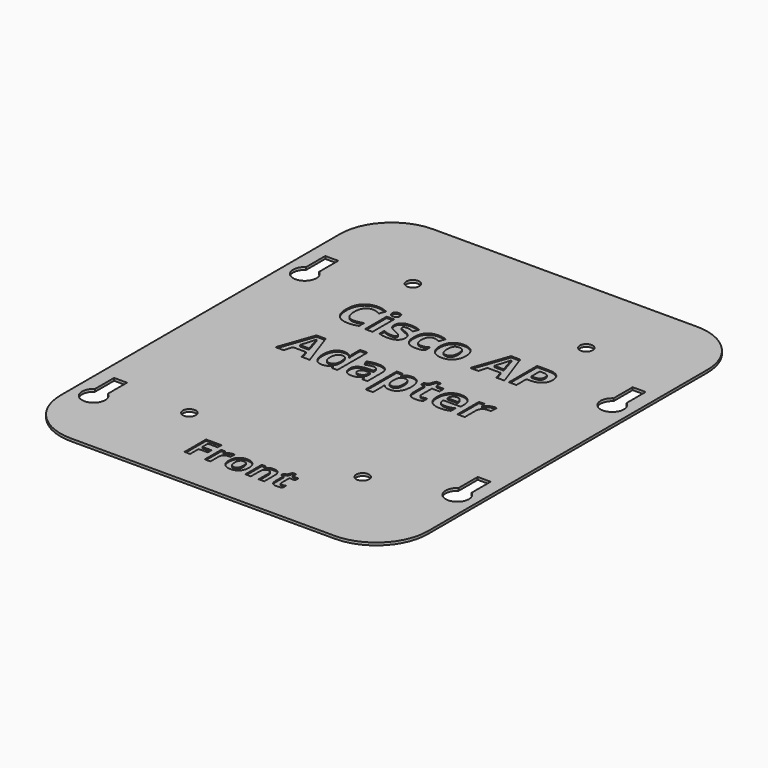
from build123d import *

# Parameters (mm, degrees)
F0_R           = 2.5
F0_W           = 2.8563935409
F0_H           = 10.4724438949
F0_TEXT_SIZE   = 19.1824959724
F0_TEXT_SIZE_2 = 14.5661450925
F1_DEPTH       = 0.5
F2_DEPTH       = 0.5


# Not quite as in the source:
# - Text() gives the source's letters only with a copy of the font that has no kerning and outlines rounded to 1/6400 em; it was checked with that copy


with BuildPart() as f1:
    # F0 (on Top) → F1 (new body)
    with BuildSketch(Plane.XY):
        with BuildLine():
            Line((51, 87.5), (-51, 87.5))
            ThreePointArc((-51, 87.5), (-65.1421356237, 81.6421356237), (-71, 67.5))
            Line((-71, 67.5), (-71, -67.5))
            ThreePointArc((-71, -67.5), (-65.1421356237, -81.6421356237), (-51, -87.5))
            Line((-51, -87.5), (51, -87.5))
            ThreePointArc((51, -87.5), (65.1421356237, -81.6421356237), (71, -67.5))
            Line((71, -67.5), (71, 67.5))
            ThreePointArc((71, 67.5), (65.1421356237, 81.6421356237), (51, 87.5))
        make_face()
        with BuildLine():
            Line((-65.5, -48.5), (-60.5, -48.5))
            Line((-60.5, -48.5), (-60.5, -57.7583426132))
            ThreePointArc((-60.5, -57.7583426132), (-63, -66), (-65.5, -57.7583426132))
            Line((-65.5, -57.7583426132), (-65.5, -48.5))
        make_face(mode=Mode.SUBTRACT)
        Polygon((-16.5223328592, -68.8772403983), (-16.5223328592, -72.9876244666), (-18.6913229018, -72.9876244666), (-18.6913229018, -62.5887624467), (-12.7305832148, -62.5887624467), (-12.7305832148, -64.3958748222), (-16.5223328592, -64.3958748222), (-16.5223328592, -67.0769559033), (-12.9945945946, -67.0769559033), (-12.9945945946, -68.8772403983), align=None, mode=Mode.SUBTRACT)
        with BuildLine():
            add(Edge.make_bspline(
                [(-7.7974395448, -65.2960170697), (-7.1681365576, -64.8874822191), (-6.4284495021, -64.8874822191)],
                knots=[0, 0, 0, 1, 1, 1], degree=2))
            add(Edge.make_bspline(
                [(-6.4284495021, -64.8874822191), (-5.986913229, -64.8874822191), (-5.6955903272, -64.9512091038)],
                knots=[0, 0, 0, 1, 1, 1], degree=2))
            Line((-5.6955903272, -64.9512091038), (-5.8594594595, -66.9836415363))
            add(Edge.make_bspline(
                [(-5.8594594595, -66.9836415363), (-6.1234708393, -66.913086771), (-6.4990042674, -66.913086771)],
                knots=[0, 0, 0, 1, 1, 1], degree=2))
            add(Edge.make_bspline(
                [(-6.4990042674, -66.913086771), (-7.5368421053, -66.913086771), (-8.1172119488, -67.446799431)],
                knots=[0, 0, 0, 1, 1, 1], degree=2))
            add(Edge.make_bspline(
                [(-8.1172119488, -67.446799431), (-8.6975817923, -67.980512091), (-8.6975817923, -68.9409672831)],
                knots=[0, 0, 0, 1, 1, 1], degree=2))
            Line((-8.6975817923, -68.9409672831), (-8.6975817923, -72.9876244666))
            Line((-8.6975817923, -72.9876244666), (-10.866571835, -72.9876244666))
            Line((-10.866571835, -72.9876244666), (-10.866571835, -65.0354196302))
            Line((-10.866571835, -65.0354196302), (-9.2233285917, -65.0354196302))
            Line((-9.2233285917, -65.0354196302), (-8.9024182077, -66.3736842105))
            Line((-8.9024182077, -66.3736842105), (-8.7977240398, -66.3736842105))
            add(Edge.make_bspline(
                [(-8.7977240398, -66.3736842105), (-8.426742532, -65.7045519203), (-7.7974395448, -65.2960170697)],
                knots=[0, 0, 0, 1, 1, 1], degree=2))
        make_face(mode=Mode.SUBTRACT)
        with BuildLine():
            add(Edge.make_bspline(
                [(2.5046941679, -66.8140825036), (2.973541963, -67.7460881935), (2.973541963, -68.9978662873)],
                knots=[0, 0, 0, 1, 1, 1], degree=2))
            add(Edge.make_bspline(
                [(2.973541963, -68.9978662873), (2.973541963, -70.9392603129), (1.9493598862, -72.0351351351)],
                knots=[0, 0, 0, 1, 1, 1], degree=2))
            add(Edge.make_bspline(
                [(1.9493598862, -72.0351351351), (0.9251778094, -73.1310099573), (-0.9024182077, -73.1310099573)],
                knots=[0, 0, 0, 1, 1, 1], degree=2))
            add(Edge.make_bspline(
                [(-0.9024182077, -73.1310099573), (-2.0472261735, -73.1310099573), (-2.9223328592, -72.6291607397)],
                knots=[0, 0, 0, 1, 1, 1], degree=2))
            add(Edge.make_bspline(
                [(-2.9223328592, -72.6291607397), (-3.7974395448, -72.127311522), (-4.26628734, -71.1884779516)],
                knots=[0, 0, 0, 1, 1, 1], degree=2))
            add(Edge.make_bspline(
                [(-4.26628734, -71.1884779516), (-4.7351351351, -70.2496443812), (-4.7351351351, -68.9978662873)],
                knots=[0, 0, 0, 1, 1, 1], degree=2))
            add(Edge.make_bspline(
                [(-4.7351351351, -68.9978662873), (-4.7351351351, -67.0496443812), (-3.7189189189, -65.9685633001)],
                knots=[0, 0, 0, 1, 1, 1], degree=2))
            add(Edge.make_bspline(
                [(-3.7189189189, -65.9685633001), (-2.7027027027, -64.8874822191), (-0.8591749644, -64.8874822191)],
                knots=[0, 0, 0, 1, 1, 1], degree=2))
            add(Edge.make_bspline(
                [(-0.8591749644, -64.8874822191), (0.2856330014, -64.8874822191), (1.1607396871, -65.3847795164)],
                knots=[0, 0, 0, 1, 1, 1], degree=2))
            add(Edge.make_bspline(
                [(1.1607396871, -65.3847795164), (2.0358463727, -65.8820768137), (2.5046941679, -66.8140825036)],
                knots=[0, 0, 0, 1, 1, 1], degree=2))
        make_face(mode=Mode.SUBTRACT)
        with Locations((-33.5, -52.1582150757)):
            Circle(F0_R, mode=Mode.SUBTRACT)
        with BuildLine():
            Line((12.106970128, -67.8029871977), (12.106970128, -72.9876244666))
            Line((12.106970128, -72.9876244666), (9.9379800853, -72.9876244666))
            Line((9.9379800853, -72.9876244666), (9.9379800853, -68.3423897582))
            add(Edge.make_bspline(
                [(9.9379800853, -68.3423897582), (9.9379800853, -67.4820768137), (9.6318634424, -67.0519203414)],
                knots=[0, 0, 0, 1, 1, 1], degree=2))
            add(Edge.make_bspline(
                [(9.6318634424, -67.0519203414), (9.3257467994, -66.6217638691), (8.6566145092, -66.6217638691)],
                knots=[0, 0, 0, 1, 1, 1], degree=2))
            add(Edge.make_bspline(
                [(8.6566145092, -66.6217638691), (7.746230441, -66.6217638691), (7.3411095306, -67.2294452347)],
                knots=[0, 0, 0, 1, 1, 1], degree=2))
            add(Edge.make_bspline(
                [(7.3411095306, -67.2294452347), (6.9359886202, -67.8371266003), (6.9359886202, -69.2459459459)],
                knots=[0, 0, 0, 1, 1, 1], degree=2))
            Line((6.9359886202, -69.2459459459), (6.9359886202, -72.9876244666))
            Line((6.9359886202, -72.9876244666), (4.7669985775, -72.9876244666))
            Line((4.7669985775, -72.9876244666), (4.7669985775, -65.0354196302))
            Line((4.7669985775, -65.0354196302), (6.4238975818, -65.0354196302))
            Line((6.4238975818, -65.0354196302), (6.7152204836, -66.0527738265))
            Line((6.7152204836, -66.0527738265), (6.8358463727, -66.0527738265))
            add(Edge.make_bspline(
                [(6.8358463727, -66.0527738265), (7.2, -65.4769559033), (7.8361308677, -65.1822190612)],
                knots=[0, 0, 0, 1, 1, 1], degree=2))
            add(Edge.make_bspline(
                [(7.8361308677, -65.1822190612), (8.4722617354, -64.8874822191), (9.2825035562, -64.8874822191)],
                knots=[0, 0, 0, 1, 1, 1], degree=2))
            add(Edge.make_bspline(
                [(9.2825035562, -64.8874822191), (10.6708392603, -64.8874822191), (11.3889046942, -65.6374110953)],
                knots=[0, 0, 0, 1, 1, 1], degree=2))
            add(Edge.make_bspline(
                [(11.3889046942, -65.6374110953), (12.106970128, -66.3873399716), (12.106970128, -67.8029871977)],
                knots=[0, 0, 0, 1, 1, 1], degree=2))
        make_face(mode=Mode.SUBTRACT)
        with BuildLine():
            add(Edge.make_bspline(
                [(17.0025604552, -71.180512091), (17.2620199147, -71.4012802276), (17.6899004267, -71.4012802276)],
                knots=[0, 0, 0, 1, 1, 1], degree=2))
            add(Edge.make_bspline(
                [(17.6899004267, -71.4012802276), (18.2588904694, -71.4012802276), (19.0554765292, -71.153200569)],
                knots=[0, 0, 0, 1, 1, 1], degree=2))
            Line((19.0554765292, -71.153200569), (19.0554765292, -72.76685633))
            add(Edge.make_bspline(
                [(19.0554765292, -72.76685633), (18.2452347084, -73.1310099573), (17.0640113798, -73.1310099573)],
                knots=[0, 0, 0, 1, 1, 1], degree=2))
            add(Edge.make_bspline(
                [(17.0640113798, -73.1310099573), (15.7621621622, -73.1310099573), (15.1681365576, -72.4721194879)],
                knots=[0, 0, 0, 1, 1, 1], degree=2))
            add(Edge.make_bspline(
                [(15.1681365576, -72.4721194879), (14.5741109531, -71.8132290185), (14.5741109531, -70.4977240398)],
                knots=[0, 0, 0, 1, 1, 1], degree=2))
            Line((14.5741109531, -70.4977240398), (14.5741109531, -66.6650071124))
            Line((14.5741109531, -66.6650071124), (13.5362731152, -66.6650071124))
            Line((13.5362731152, -66.6650071124), (13.5362731152, -65.7477951636))
            Line((13.5362731152, -65.7477951636), (14.7311522048, -65.0217638691))
            Line((14.7311522048, -65.0217638691), (15.3570412518, -63.3421052632))
            Line((15.3570412518, -63.3421052632), (16.7431009957, -63.3421052632))
            Line((16.7431009957, -63.3421052632), (16.7431009957, -65.0354196302))
            Line((16.7431009957, -65.0354196302), (18.9689900427, -65.0354196302))
            Line((18.9689900427, -65.0354196302), (18.9689900427, -66.6650071124))
            Line((18.9689900427, -66.6650071124), (16.7431009957, -66.6650071124))
            Line((16.7431009957, -66.6650071124), (16.7431009957, -70.4977240398))
            add(Edge.make_bspline(
                [(16.7431009957, -70.4977240398), (16.7431009957, -70.9597439545), (17.0025604552, -71.180512091)],
                knots=[0, 0, 0, 1, 1, 1], degree=2))
        make_face(mode=Mode.SUBTRACT)
        with Locations((33.5, -52.1582150757)):
            Circle(F0_R, mode=Mode.SUBTRACT)
        with BuildLine():
            Line((60.6190240383, -30.5), (65.6190240383, -30.5))
            Line((65.6190240383, -30.5), (65.6190240383, -39.7583426132))
            ThreePointArc((65.6190240383, -39.7583426132), (63.1190240383, -48), (60.6190240383, -39.7583426132))
            Line((60.6190240383, -39.7583426132), (60.6190240383, -30.5))
        make_face(mode=Mode.SUBTRACT)
        Polygon((-26.764077779, -2.3995916226), (-29.8932224345, -2.3995916226), (-30.8853171481, 0.8614326927), (-35.8787606309, 0.8614326927), (-36.8708553445, -2.3995916226), (-40, -2.3995916226), (-35.1654115619, 11.3518601776), (-31.6166498071, 11.3518601776), align=None, mode=Mode.SUBTRACT)
        with BuildLine():
            add(Edge.make_bspline(
                [(-18.9801805852, -1.0418305796), (-19.9542917088, -2.5884193174), (-21.9504701959, -2.5884193174)],
                knots=[0, 0, 0, 1, 1, 1], degree=2))
            add(Edge.make_bspline(
                [(-21.9504701959, -2.5884193174), (-23.7937881683, -2.5884193174), (-24.8473268143, -1.1542280169)],
                knots=[0, 0, 0, 1, 1, 1], degree=2))
            add(Edge.make_bspline(
                [(-24.8473268143, -1.1542280169), (-25.9008654603, 0.2799632835), (-25.9008654603, 2.8186467349)],
                knots=[0, 0, 0, 1, 1, 1], degree=2))
            add(Edge.make_bspline(
                [(-25.9008654603, 2.8186467349), (-25.9008654603, 5.3932973662), (-24.8293432243, 6.8304859316)],
                knots=[0, 0, 0, 1, 1, 1], degree=2))
            add(Edge.make_bspline(
                [(-24.8293432243, 6.8304859316), (-23.7578209883, 8.267674497), (-21.8755385711, 8.267674497)],
                knots=[0, 0, 0, 1, 1, 1], degree=2))
            add(Edge.make_bspline(
                [(-21.8755385711, 8.267674497), (-19.8973436739, 8.267674497), (-18.8572927204, 6.7330748192)],
                knots=[0, 0, 0, 1, 1, 1], degree=2))
            Line((-18.8572927204, 6.7330748192), (-18.7643775055, 6.7330748192))
            add(Edge.make_bspline(
                [(-18.7643775055, 6.7330748192), (-18.9801805852, 7.9050054325), (-18.9801805852, 8.8221685212)],
                knots=[0, 0, 0, 1, 1, 1], degree=2))
            Line((-18.9801805852, 8.8221685212), (-18.9801805852, 12.1761080514))
            Line((-18.9801805852, 12.1761080514), (-16.1147952493, 12.1761080514))
            Line((-16.1147952493, 12.1761080514), (-16.1147952493, -2.3995916226))
            Line((-16.1147952493, -2.3995916226), (-18.3057959612, -2.3995916226))
            Line((-18.3057959612, -2.3995916226), (-18.8572927204, -1.0418305796))
            Line((-18.8572927204, -1.0418305796), (-18.9801805852, -1.0418305796))
        make_face(mode=Mode.SUBTRACT)
        with BuildLine():
            Line((-4.4824098011, -2.3995916226), (-6.4755910232, -2.3995916226))
            Line((-6.4755910232, -2.3995916226), (-7.0300850474, -0.9758907497))
            Line((-7.0300850474, -0.9758907497), (-7.1050166723, -0.9758907497))
            add(Edge.make_bspline(
                [(-7.1050166723, -0.9758907497), (-7.8243602713, -1.8840620434), (-8.5886628452, -2.2362406804)],
                knots=[0, 0, 0, 1, 1, 1], degree=2))
            add(Edge.make_bspline(
                [(-8.5886628452, -2.2362406804), (-9.3529654191, -2.5884193174), (-10.5788468023, -2.5884193174)],
                knots=[0, 0, 0, 1, 1, 1], degree=2))
            add(Edge.make_bspline(
                [(-10.5788468023, -2.5884193174), (-12.0864710951, -2.5884193174), (-12.9526806789, -1.7252069986)],
                knots=[0, 0, 0, 1, 1, 1], degree=2))
            add(Edge.make_bspline(
                [(-12.9526806789, -1.7252069986), (-13.8188902626, -0.8619946799), (-13.8188902626, 0.7295530329)],
                knots=[0, 0, 0, 1, 1, 1], degree=2))
            add(Edge.make_bspline(
                [(-13.8188902626, 0.7295530329), (-13.8188902626, 2.3960323705), (-12.6529541793, 3.1873103293)],
                knots=[0, 0, 0, 1, 1, 1], degree=2))
            add(Edge.make_bspline(
                [(-12.6529541793, 3.1873103293), (-11.487018096, 3.9785882882), (-9.1371623394, 4.0625117081)],
                knots=[0, 0, 0, 1, 1, 1], degree=2))
            Line((-9.1371623394, 4.0625117081), (-7.317822487, 4.119459743))
            Line((-7.317822487, 4.119459743), (-7.317822487, 4.5780412873))
            add(Edge.make_bspline(
                [(-7.317822487, 4.5780412873), (-7.317822487, 6.169589), (-8.9483346446, 6.169589)],
                knots=[0, 0, 0, 1, 1, 1], degree=2))
            add(Edge.make_bspline(
                [(-8.9483346446, 6.169589), (-10.2041886778, 6.169589), (-11.9006406654, 5.4112809561)],
                knots=[0, 0, 0, 1, 1, 1], degree=2))
            Line((-11.9006406654, 5.4112809561), (-12.844779139, 7.3415196134))
            add(Edge.make_bspline(
                [(-12.844779139, 7.3415196134), (-11.0374283466, 8.288655352), (-8.8374358398, 8.288655352)],
                knots=[0, 0, 0, 1, 1, 1], degree=2))
            add(Edge.make_bspline(
                [(-8.8374358398, 8.288655352), (-6.7303585478, 8.288655352), (-5.6063841744, 7.3699936308)],
                knots=[0, 0, 0, 1, 1, 1], degree=2))
            add(Edge.make_bspline(
                [(-5.6063841744, 7.3699936308), (-4.4824098011, 6.4513319096), (-4.4824098011, 4.5780412873)],
                knots=[0, 0, 0, 1, 1, 1], degree=2))
            Line((-4.4824098011, 4.5780412873), (-4.4824098011, -2.3995916226))
        make_face(mode=Mode.SUBTRACT)
        with BuildLine():
            add(Edge.make_bspline(
                [(-30.933273388, 34.8908808213), (-31.7095650219, 35.1621333034), (-32.4588812708, 35.1621333034)],
                knots=[0, 0, 0, 1, 1, 1], degree=2))
            add(Edge.make_bspline(
                [(-32.4588812708, 35.1621333034), (-34.0983852235, 35.1621333034), (-34.9975647222, 33.9302573901)],
                knots=[0, 0, 0, 1, 1, 1], degree=2))
            add(Edge.make_bspline(
                [(-34.9975647222, 33.9302573901), (-35.8967442209, 32.6983814769), (-35.8967442209, 30.4983889701)],
                knots=[0, 0, 0, 1, 1, 1], degree=2))
            add(Edge.make_bspline(
                [(-35.8967442209, 30.4983889701), (-35.8967442209, 25.9185680566), (-32.4588812708, 25.9185680566)],
                knots=[0, 0, 0, 1, 1, 1], degree=2))
            add(Edge.make_bspline(
                [(-32.4588812708, 25.9185680566), (-31.0171968079, 25.9185680566), (-28.9670675509, 26.6379116556)],
                knots=[0, 0, 0, 1, 1, 1], degree=2))
            Line((-28.9670675509, 26.6379116556), (-28.9670675509, 24.2041324791))
            add(Edge.make_bspline(
                [(-28.9670675509, 24.2041324791), (-30.6515304784, 23.4997752051), (-32.7316323854, 23.4997752051)],
                knots=[0, 0, 0, 1, 1, 1], degree=2))
            add(Edge.make_bspline(
                [(-32.7316323854, 23.4997752051), (-35.7199055862, 23.4997752051), (-37.3024615039, 25.3131205275)],
                knots=[0, 0, 0, 1, 1, 1], degree=2))
            add(Edge.make_bspline(
                [(-37.3024615039, 25.3131205275), (-38.8850174216, 27.1264658499), (-38.8850174216, 30.51637256)],
                knots=[0, 0, 0, 1, 1, 1], degree=2))
            add(Edge.make_bspline(
                [(-38.8850174216, 30.51637256), (-38.8850174216, 32.653422502), (-38.1072271552, 34.2599565397)],
                knots=[0, 0, 0, 1, 1, 1], degree=2))
            add(Edge.make_bspline(
                [(-38.1072271552, 34.2599565397), (-37.3294368888, 35.8664905773), (-35.8727661009, 36.7222097336)],
                knots=[0, 0, 0, 1, 1, 1], degree=2))
            add(Edge.make_bspline(
                [(-35.8727661009, 36.7222097336), (-34.416095313, 37.5779288899), (-32.4588812708, 37.5779288899)],
                knots=[0, 0, 0, 1, 1, 1], degree=2))
            add(Edge.make_bspline(
                [(-32.4588812708, 37.5779288899), (-30.4657000487, 37.5779288899), (-28.4515379716, 36.6158068263)],
                knots=[0, 0, 0, 1, 1, 1], degree=2))
            Line((-28.4515379716, 36.6158068263), (-29.3866846503, 34.2539620097))
            add(Edge.make_bspline(
                [(-29.3866846503, 34.2539620097), (-30.1569817541, 34.6196283391), (-30.933273388, 34.8908808213)],
                knots=[0, 0, 0, 1, 1, 1], degree=2))
        make_face(mode=Mode.SUBTRACT)
        with Locations((-24.8503240793, 28.9248248473)):
            Rectangle(F0_W, F0_H, mode=Mode.SUBTRACT)
        with BuildLine():
            add(Edge.make_bspline(
                [(-24.8458281818, 35.4618598029), (-26.4014087145, 35.4618598029), (-26.4014087145, 36.8675770859)],
                knots=[0, 0, 0, 1, 1, 1], degree=2))
            add(Edge.make_bspline(
                [(-26.4014087145, 36.8675770859), (-26.4014087145, 38.2643025739), (-24.8458281818, 38.2643025739)],
                knots=[0, 0, 0, 1, 1, 1], degree=2))
            add(Edge.make_bspline(
                [(-24.8458281818, 38.2643025739), (-23.290247649, 38.2643025739), (-23.290247649, 36.8675770859)],
                knots=[0, 0, 0, 1, 1, 1], degree=2))
            add(Edge.make_bspline(
                [(-23.290247649, 36.8675770859), (-23.290247649, 36.2021842569), (-23.678393466, 35.8320220299)],
                knots=[0, 0, 0, 1, 1, 1], degree=2))
            add(Edge.make_bspline(
                [(-23.678393466, 35.8320220299), (-24.0665392829, 35.4618598029), (-24.8458281818, 35.4618598029)],
                knots=[0, 0, 0, 1, 1, 1], degree=2))
        make_face(mode=Mode.SUBTRACT)
        with BuildLine():
            add(Edge.make_bspline(
                [(-13.3902813683, 28.138042786), (-13.1175302536, 27.5760555993), (-13.1175302536, 26.7997639654)],
                knots=[0, 0, 0, 1, 1, 1], degree=2))
            add(Edge.make_bspline(
                [(-13.1175302536, 26.7997639654), (-13.1175302536, 25.1872353977), (-14.2370087295, 24.3435053014)],
                knots=[0, 0, 0, 1, 1, 1], degree=2))
            add(Edge.make_bspline(
                [(-14.2370087295, 24.3435053014), (-15.3564872054, 23.4997752051), (-17.5864523622, 23.4997752051)],
                knots=[0, 0, 0, 1, 1, 1], degree=2))
            add(Edge.make_bspline(
                [(-17.5864523622, 23.4997752051), (-18.7284103256, 23.4997752051), (-19.5346746094, 23.6556329849)],
                knots=[0, 0, 0, 1, 1, 1], degree=2))
            add(Edge.make_bspline(
                [(-19.5346746094, 23.6556329849), (-20.3409388933, 23.8114907647), (-21.0422989023, 24.1112172642)],
                knots=[0, 0, 0, 1, 1, 1], degree=2))
            Line((-21.0422989023, 24.1112172642), (-21.0422989023, 26.4700648159))
            add(Edge.make_bspline(
                [(-21.0422989023, 26.4700648159), (-20.2480236784, 26.0954066914), (-19.2499344348, 25.8421377993)],
                knots=[0, 0, 0, 1, 1, 1], degree=2))
            add(Edge.make_bspline(
                [(-19.2499344348, 25.8421377993), (-18.2518451913, 25.5888689071), (-17.4935371474, 25.5888689071)],
                knots=[0, 0, 0, 1, 1, 1], degree=2))
            add(Edge.make_bspline(
                [(-17.4935371474, 25.5888689071), (-15.9379566146, 25.5888689071), (-15.9379566146, 26.4880484058)],
                knots=[0, 0, 0, 1, 1, 1], degree=2))
            add(Edge.make_bspline(
                [(-15.9379566146, 26.4880484058), (-15.9379566146, 26.8267393503), (-16.1447678993, 27.0380465325)],
                knots=[0, 0, 0, 1, 1, 1], degree=2))
            add(Edge.make_bspline(
                [(-16.1447678993, 27.0380465325), (-16.351579184, 27.2493537147), (-16.8566183358, 27.5161102994)],
                knots=[0, 0, 0, 1, 1, 1], degree=2))
            add(Edge.make_bspline(
                [(-16.8566183358, 27.5161102994), (-17.3616574875, 27.782866884), (-18.2038889513, 28.1365441535)],
                knots=[0, 0, 0, 1, 1, 1], degree=2))
            add(Edge.make_bspline(
                [(-18.2038889513, 28.1365441535), (-19.4117867446, 28.6430819377), (-19.9797684613, 29.0746880971)],
                knots=[0, 0, 0, 1, 1, 1], degree=2))
            add(Edge.make_bspline(
                [(-19.9797684613, 29.0746880971), (-20.547750178, 29.5062942565), (-20.8040163351, 30.0637855457)],
                knots=[0, 0, 0, 1, 1, 1], degree=2))
            add(Edge.make_bspline(
                [(-20.8040163351, 30.0637855457), (-21.0602824922, 30.6212768349), (-21.0602824922, 31.4335356487)],
                knots=[0, 0, 0, 1, 1, 1], degree=2))
            add(Edge.make_bspline(
                [(-21.0602824922, 31.4335356487), (-21.0602824922, 32.8302611367), (-19.9797684613, 33.5930650781)],
                knots=[0, 0, 0, 1, 1, 1], degree=2))
            add(Edge.make_bspline(
                [(-19.9797684613, 33.5930650781), (-18.8992544303, 34.3558690195), (-16.9120677382, 34.3558690195)],
                knots=[0, 0, 0, 1, 1, 1], degree=2))
            add(Edge.make_bspline(
                [(-16.9120677382, 34.3558690195), (-15.0207935259, 34.3558690195), (-13.2314263235, 33.5316211457)],
                knots=[0, 0, 0, 1, 1, 1], degree=2))
            Line((-13.2314263235, 33.5316211457), (-14.0916413772, 31.4725000937))
            add(Edge.make_bspline(
                [(-14.0916413772, 31.4725000937), (-14.8799220711, 31.8081937732), (-15.5632984901, 32.0239968529)],
                knots=[0, 0, 0, 1, 1, 1], degree=2))
            add(Edge.make_bspline(
                [(-15.5632984901, 32.0239968529), (-16.2466749091, 32.2397999326), (-16.9600239781, 32.2397999326)],
                knots=[0, 0, 0, 1, 1, 1], degree=2))
            add(Edge.make_bspline(
                [(-16.9600239781, 32.2397999326), (-18.2248698063, 32.2397999326), (-18.2248698063, 31.5564235135)],
                knots=[0, 0, 0, 1, 1, 1], degree=2))
            add(Edge.make_bspline(
                [(-18.2248698063, 31.5564235135), (-18.2248698063, 31.1727735941), (-17.8172417669, 30.8910306845)],
                knots=[0, 0, 0, 1, 1, 1], degree=2))
            add(Edge.make_bspline(
                [(-17.8172417669, 30.8910306845), (-17.4096137275, 30.6092877749), (-16.0308718295, 30.0577910157)],
                knots=[0, 0, 0, 1, 1, 1], degree=2))
            add(Edge.make_bspline(
                [(-16.0308718295, 30.0577910157), (-14.8049904462, 29.5602450264), (-14.2340114645, 29.1301374995)],
                knots=[0, 0, 0, 1, 1, 1], degree=2))
            add(Edge.make_bspline(
                [(-14.2340114645, 29.1301374995), (-13.6630324829, 28.7000299726), (-13.3902813683, 28.138042786)],
                knots=[0, 0, 0, 1, 1, 1], degree=2))
        make_face(mode=Mode.SUBTRACT)
        with BuildLine():
            add(Edge.make_bspline(
                [(-4.8540706605, 23.6691206774), (-5.5614251995, 23.4997752051), (-6.637443333, 23.4997752051)],
                knots=[0, 0, 0, 1, 1, 1], degree=2))
            add(Edge.make_bspline(
                [(-6.637443333, 23.4997752051), (-11.5259825409, 23.4997752051), (-11.5259825409, 28.8678768124)],
                knots=[0, 0, 0, 1, 1, 1], degree=2))
            add(Edge.make_bspline(
                [(-11.5259825409, 28.8678768124), (-11.5259825409, 31.5384399236), (-10.1966955153, 32.9471544715)],
                knots=[0, 0, 0, 1, 1, 1], degree=2))
            add(Edge.make_bspline(
                [(-10.1966955153, 32.9471544715), (-8.8674084898, 34.3558690195), (-6.3856730733, 34.3558690195)],
                knots=[0, 0, 0, 1, 1, 1], degree=2))
            add(Edge.make_bspline(
                [(-6.3856730733, 34.3558690195), (-4.5693304859, 34.3558690195), (-3.124648758, 33.6455172155)],
                knots=[0, 0, 0, 1, 1, 1], degree=2))
            Line((-3.124648758, 33.6455172155), (-3.9698774868, 31.4335356487))
            add(Edge.make_bspline(
                [(-3.9698774868, 31.4335356487), (-4.6442621108, 31.7062867633), (-5.2242328875, 31.8801281331)],
                knots=[0, 0, 0, 1, 1, 1], degree=2))
            add(Edge.make_bspline(
                [(-5.2242328875, 31.8801281331), (-5.8042036642, 32.0539695028), (-6.3856730733, 32.0539695028)],
                knots=[0, 0, 0, 1, 1, 1], degree=2))
            add(Edge.make_bspline(
                [(-6.3856730733, 32.0539695028), (-8.6156382301, 32.0539695028), (-8.6156382301, 28.8858604024)],
                knots=[0, 0, 0, 1, 1, 1], degree=2))
            add(Edge.make_bspline(
                [(-8.6156382301, 28.8858604024), (-8.6156382301, 25.8136637818), (-6.3856730733, 25.8136637818)],
                knots=[0, 0, 0, 1, 1, 1], degree=2))
            add(Edge.make_bspline(
                [(-6.3856730733, 25.8136637818), (-5.5614251995, 25.8136637818), (-4.858566558, 26.033962759)],
                knots=[0, 0, 0, 1, 1, 1], degree=2))
            add(Edge.make_bspline(
                [(-4.858566558, 26.033962759), (-4.1557079165, 26.2542617362), (-3.4543479075, 26.7248323405)],
                knots=[0, 0, 0, 1, 1, 1], degree=2))
            Line((-3.4543479075, 26.7248323405), (-3.4543479075, 24.279064104))
            add(Edge.make_bspline(
                [(-3.4543479075, 24.279064104), (-4.1467161215, 23.8384661496), (-4.8540706605, 23.6691206774)],
                knots=[0, 0, 0, 1, 1, 1], degree=2))
        make_face(mode=Mode.SUBTRACT)
        with BuildLine():
            Line((-65.5, 53.5), (-60.5, 53.5))
            Line((-60.5, 53.5), (-60.5, 44.2416573868))
            ThreePointArc((-60.5, 44.2416573868), (-63, 36), (-65.5, 44.2416573868))
            Line((-65.5, 44.2416573868), (-65.5, 53.5))
        make_face(mode=Mode.SUBTRACT)
        with Locations((-33.5, 55.8417849243)):
            Circle(F0_R, mode=Mode.SUBTRACT)
        with BuildLine():
            add(Edge.make_bspline(
                [(6.3467086284, -1.9410100783), (5.4385373347, -2.5884193174), (4.2126559514, -2.5884193174)],
                knots=[0, 0, 0, 1, 1, 1], degree=2))
            add(Edge.make_bspline(
                [(4.2126559514, -2.5884193174), (2.3663407141, -2.5884193174), (1.3172979656, -1.2486418643)],
                knots=[0, 0, 0, 1, 1, 1], degree=2))
            Line((1.3172979656, -1.2486418643), (1.1674347158, -1.2486418643))
            add(Edge.make_bspline(
                [(1.1674347158, -1.2486418643), (1.3172979656, -2.5584466674), (1.3172979656, -2.7652579521)],
                knots=[0, 0, 0, 1, 1, 1], degree=2))
            Line((1.3172979656, -2.7652579521), (1.3172979656, -7.009385186))
            Line((1.3172979656, -7.009385186), (-1.5390955753, -7.009385186))
            Line((-1.5390955753, -7.009385186), (-1.5390955753, 8.0728522723))
            Line((-1.5390955753, 8.0728522723), (0.7837847964, 8.0728522723))
            Line((0.7837847964, 8.0728522723), (1.1854183058, 6.7150912293))
            Line((1.1854183058, 6.7150912293), (1.3172979656, 6.7150912293))
            add(Edge.make_bspline(
                [(1.3172979656, 6.7150912293), (2.3213817392, 8.267674497), (4.2875875763, 8.267674497)],
                knots=[0, 0, 0, 1, 1, 1], degree=2))
            add(Edge.make_bspline(
                [(4.2875875763, 8.267674497), (6.1428946087, 8.267674497), (7.1919373572, 6.8349818291)],
                knots=[0, 0, 0, 1, 1, 1], degree=2))
            add(Edge.make_bspline(
                [(7.1919373572, 6.8349818291), (8.2409801057, 5.4022891611), (8.2409801057, 2.8546139148)],
                knots=[0, 0, 0, 1, 1, 1], degree=2))
            add(Edge.make_bspline(
                [(8.2409801057, 2.8546139148), (8.2409801057, 1.1791427822), (7.7479300139, -0.0572290285)],
                knots=[0, 0, 0, 1, 1, 1], degree=2))
            add(Edge.make_bspline(
                [(7.7479300139, -0.0572290285), (7.2548799221, -1.2936008392), (6.3467086284, -1.9410100783)],
                knots=[0, 0, 0, 1, 1, 1], degree=2))
        make_face(mode=Mode.SUBTRACT)
        with BuildLine():
            add(Edge.make_bspline(
                [(14.1066277022, -0.0197632161), (14.4483159117, -0.3104979206), (15.0118017309, -0.3104979206)],
                knots=[0, 0, 0, 1, 1, 1], degree=2))
            add(Edge.make_bspline(
                [(15.0118017309, -0.3104979206), (15.7611179798, -0.3104979206), (16.8101607283, 0.0162039639)],
                knots=[0, 0, 0, 1, 1, 1], degree=2))
            Line((16.8101607283, 0.0162039639), (16.8101607283, -2.1088569181))
            add(Edge.make_bspline(
                [(16.8101607283, -2.1088569181), (15.7431343899, -2.5884193174), (14.1875538571, -2.5884193174)],
                knots=[0, 0, 0, 1, 1, 1], degree=2))
            add(Edge.make_bspline(
                [(14.1875538571, -2.5884193174), (12.4731182796, -2.5884193174), (11.6908321157, -1.7207111011)],
                knots=[0, 0, 0, 1, 1, 1], degree=2))
            add(Edge.make_bspline(
                [(11.6908321157, -1.7207111011), (10.9085459518, -0.8530028849), (10.9085459518, 0.8794162826)],
                knots=[0, 0, 0, 1, 1, 1], degree=2))
            Line((10.9085459518, 0.8794162826), (10.9085459518, 5.9268105354))
            Line((10.9085459518, 5.9268105354), (9.5417931138, 5.9268105354))
            Line((9.5417931138, 5.9268105354), (9.5417931138, 7.1347083287))
            Line((9.5417931138, 7.1347083287), (11.1153572365, 8.0908358623))
            Line((11.1153572365, 8.0908358623), (11.9396051103, 10.3028174291))
            Line((11.9396051103, 10.3028174291), (13.7649394927, 10.3028174291))
            Line((13.7649394927, 10.3028174291), (13.7649394927, 8.0728522723))
            Line((13.7649394927, 8.0728522723), (16.6962646585, 8.0728522723))
            Line((16.6962646585, 8.0728522723), (16.6962646585, 5.9268105354))
            Line((16.6962646585, 5.9268105354), (13.7649394927, 5.9268105354))
            Line((13.7649394927, 5.9268105354), (13.7649394927, 0.8794162826))
            add(Edge.make_bspline(
                [(13.7649394927, 0.8794162826), (13.7649394927, 0.2709714885), (14.1066277022, -0.0197632161)],
                knots=[0, 0, 0, 1, 1, 1], degree=2))
        make_face(mode=Mode.SUBTRACT)
        with BuildLine():
            add(Edge.make_bspline(
                [(25.7450076805, -2.4055861526), (24.8937844217, -2.5884193174), (23.6649057735, -2.5884193174)],
                knots=[0, 0, 0, 1, 1, 1], degree=2))
            add(Edge.make_bspline(
                [(23.6649057735, -2.5884193174), (21.1382113821, -2.5884193174), (19.7145105092, -1.1916938294)],
                knots=[0, 0, 0, 1, 1, 1], degree=2))
            add(Edge.make_bspline(
                [(19.7145105092, -1.1916938294), (18.2908096362, 0.2050316586), (18.2908096362, 2.7616986999)],
                knots=[0, 0, 0, 1, 1, 1], degree=2))
            add(Edge.make_bspline(
                [(18.2908096362, 2.7616986999), (18.2908096362, 5.3932973662), (19.6066089693, 6.8304859316)],
                knots=[0, 0, 0, 1, 1, 1], degree=2))
            add(Edge.make_bspline(
                [(19.6066089693, 6.8304859316), (20.9224083024, 8.267674497), (23.2452886741, 8.267674497)],
                knots=[0, 0, 0, 1, 1, 1], degree=2))
            add(Edge.make_bspline(
                [(23.2452886741, 8.267674497), (25.4632647709, 8.267674497), (26.6996365816, 7.0043273013)],
                knots=[0, 0, 0, 1, 1, 1], degree=2))
            add(Edge.make_bspline(
                [(26.6996365816, 7.0043273013), (27.9360083923, 5.7409801057), (27.9360083923, 3.5110149489)],
                knots=[0, 0, 0, 1, 1, 1], degree=2))
            Line((27.9360083923, 3.5110149489), (27.9360083923, 2.1232812559))
            Line((27.9360083923, 2.1232812559), (21.183170357, 2.1232812559))
            add(Edge.make_bspline(
                [(21.183170357, 2.1232812559), (21.231126597, 0.9063916676), (21.905511221, 0.2230152486)],
                knots=[0, 0, 0, 1, 1, 1], degree=2))
            add(Edge.make_bspline(
                [(21.905511221, 0.2230152486), (22.579895845, -0.4603611704), (23.7967854333, -0.4603611704)],
                knots=[0, 0, 0, 1, 1, 1], degree=2))
            add(Edge.make_bspline(
                [(23.7967854333, -0.4603611704), (24.7439211719, -0.4603611704), (25.5861526357, -0.2640403132)],
                knots=[0, 0, 0, 1, 1, 1], degree=2))
            add(Edge.make_bspline(
                [(25.5861526357, -0.2640403132), (26.4283840995, -0.067719456), (27.3455471882, 0.3638867034)],
                knots=[0, 0, 0, 1, 1, 1], degree=2))
            Line((27.3455471882, 0.3638867034), (27.3455471882, -1.8480948634))
            add(Edge.make_bspline(
                [(27.3455471882, -1.8480948634), (26.5962309393, -2.2227529879), (25.7450076805, -2.4055861526)],
                knots=[0, 0, 0, 1, 1, 1], degree=2))
        make_face(mode=Mode.SUBTRACT)
        with BuildLine():
            add(Edge.make_bspline(
                [(34.3007006107, 7.7296654303), (35.129444382, 8.267674497), (36.1035555056, 8.267674497)],
                knots=[0, 0, 0, 1, 1, 1], degree=2))
            add(Edge.make_bspline(
                [(36.1035555056, 8.267674497), (36.6850249148, 8.267674497), (37.0686748342, 8.1837510771)],
                knots=[0, 0, 0, 1, 1, 1], degree=2))
            Line((37.0686748342, 8.1837510771), (36.8528717545, 5.507193436))
            add(Edge.make_bspline(
                [(36.8528717545, 5.507193436), (36.505189015, 5.6001086509), (36.0106402907, 5.6001086509)],
                knots=[0, 0, 0, 1, 1, 1], degree=2))
            add(Edge.make_bspline(
                [(36.0106402907, 5.6001086509), (34.6438874527, 5.6001086509), (33.8795848788, 4.8972500094)],
                knots=[0, 0, 0, 1, 1, 1], degree=2))
            add(Edge.make_bspline(
                [(33.8795848788, 4.8972500094), (33.1152823049, 4.1943913679), (33.1152823049, 2.9295455397)],
                knots=[0, 0, 0, 1, 1, 1], degree=2))
            Line((33.1152823049, 2.9295455397), (33.1152823049, -2.3995916226))
            Line((33.1152823049, -2.3995916226), (30.258888764, -2.3995916226))
            Line((30.258888764, -2.3995916226), (30.258888764, 8.0728522723))
            Line((30.258888764, 8.0728522723), (32.4229140909, 8.0728522723))
            Line((32.4229140909, 8.0728522723), (32.8455284553, 6.3104604548))
            Line((32.8455284553, 6.3104604548), (32.9834026451, 6.3104604548))
            add(Edge.make_bspline(
                [(32.9834026451, 6.3104604548), (33.4719568394, 7.1916563636), (34.3007006107, 7.7296654303)],
                knots=[0, 0, 0, 1, 1, 1], degree=2))
        make_face(mode=Mode.SUBTRACT)
        with BuildLine():
            add(Edge.make_bspline(
                [(7.8723165112, 31.8186842007), (8.4897531003, 30.5913041849), (8.4897531003, 28.9428084373)],
                knots=[0, 0, 0, 1, 1, 1], degree=2))
            add(Edge.make_bspline(
                [(8.4897531003, 28.9428084373), (8.4897531003, 26.386141396), (7.1409838522, 24.9429583006)],
                knots=[0, 0, 0, 1, 1, 1], degree=2))
            add(Edge.make_bspline(
                [(7.1409838522, 24.9429583006), (5.7922146042, 23.4997752051), (3.3854108126, 23.4997752051)],
                knots=[0, 0, 0, 1, 1, 1], degree=2))
            add(Edge.make_bspline(
                [(3.3854108126, 23.4997752051), (1.8777865198, 23.4997752051), (0.725338129, 24.1606721367)],
                knots=[0, 0, 0, 1, 1, 1], degree=2))
            add(Edge.make_bspline(
                [(0.725338129, 24.1606721367), (-0.4271102619, 24.8215690682), (-1.044546851, 26.0579408789)],
                knots=[0, 0, 0, 1, 1, 1], degree=2))
            add(Edge.make_bspline(
                [(-1.044546851, 26.0579408789), (-1.6619834401, 27.2943126897), (-1.6619834401, 28.9428084373)],
                knots=[0, 0, 0, 1, 1, 1], degree=2))
            add(Edge.make_bspline(
                [(-1.6619834401, 28.9428084373), (-1.6619834401, 31.5084672736), (-0.3237046195, 32.9321681466)],
                knots=[0, 0, 0, 1, 1, 1], degree=2))
            add(Edge.make_bspline(
                [(-0.3237046195, 32.9321681466), (1.014574201, 34.3558690195), (3.4423588476, 34.3558690195)],
                knots=[0, 0, 0, 1, 1, 1], degree=2))
            add(Edge.make_bspline(
                [(3.4423588476, 34.3558690195), (4.9499831404, 34.3558690195), (6.1024315312, 33.700966618)],
                knots=[0, 0, 0, 1, 1, 1], degree=2))
            add(Edge.make_bspline(
                [(6.1024315312, 33.700966618), (7.2548799221, 33.0460642164), (7.8723165112, 31.8186842007)],
                knots=[0, 0, 0, 1, 1, 1], degree=2))
        make_face(mode=Mode.SUBTRACT)
        Polygon((27.5733393279, 23.6886028999), (24.4441946724, 23.6886028999), (23.4520999588, 26.9496272152), (18.458656476, 26.9496272152), (17.4665617624, 23.6886028999), (14.3374171069, 23.6886028999), (19.1720055449, 37.4400547001), (22.7207672998, 37.4400547001), align=None, mode=Mode.SUBTRACT)
        with BuildLine():
            add(Edge.make_bspline(
                [(37.4598179162, 36.3100857967), (38.7561350268, 35.2370649283), (38.7561350268, 33.1120040463)],
                knots=[0, 0, 0, 1, 1, 1], degree=2))
            add(Edge.make_bspline(
                [(38.7561350268, 33.1120040463), (38.7561350268, 30.9000224795), (37.3743958638, 29.7295904987)],
                knots=[0, 0, 0, 1, 1, 1], degree=2))
            add(Edge.make_bspline(
                [(37.3743958638, 29.7295904987), (35.9926567008, 28.5591585179), (33.4449814544, 28.5591585179)],
                knots=[0, 0, 0, 1, 1, 1], degree=2))
            Line((33.4449814544, 28.5591585179), (32.2011164812, 28.5591585179))
            Line((32.2011164812, 28.5591585179), (32.2011164812, 23.6886028999))
            Line((32.2011164812, 23.6886028999), (29.2967667004, 23.6886028999))
            Line((29.2967667004, 23.6886028999), (29.2967667004, 37.3831066652))
            Line((29.2967667004, 37.3831066652), (33.6697763291, 37.3831066652))
            add(Edge.make_bspline(
                [(33.6697763291, 37.3831066652), (36.1635008055, 37.3831066652), (37.4598179162, 36.3100857967)],
                knots=[0, 0, 0, 1, 1, 1], degree=2))
        make_face(mode=Mode.SUBTRACT)
        with BuildLine():
            Line((60.5, 44.5), (65.5, 44.5))
            Line((65.5, 44.5), (65.5, 35.2416573868))
            ThreePointArc((65.5, 35.2416573868), (63, 27), (60.5, 35.2416573868))
            Line((60.5, 35.2416573868), (60.5, 44.5))
        make_face(mode=Mode.SUBTRACT)
        with Locations((33.5, 55.8417849243)):
            Circle(F0_R, mode=Mode.SUBTRACT)
        with BuildLine():
            add(Edge.make_bspline(
                [(1.754898655, 31.2806751339), (1.2483608707, 30.5073807651), (1.2483608707, 28.9428084373)],
                knots=[0, 0, 0, 1, 1, 1], degree=2))
            add(Edge.make_bspline(
                [(1.2483608707, 28.9428084373), (1.2483608707, 27.3872279045), (1.7593945525, 26.5914540482)],
                knots=[0, 0, 0, 1, 1, 1], degree=2))
            add(Edge.make_bspline(
                [(1.7593945525, 26.5914540482), (2.2704282342, 25.7956801918), (3.4213779926, 25.7956801918)],
                knots=[0, 0, 0, 1, 1, 1], degree=2))
            add(Edge.make_bspline(
                [(3.4213779926, 25.7956801918), (4.5663332209, 25.7956801918), (5.0668764752, 26.5869581507)],
                knots=[0, 0, 0, 1, 1, 1], degree=2))
            add(Edge.make_bspline(
                [(5.0668764752, 26.5869581507), (5.5674197295, 27.3782361096), (5.5674197295, 28.9428084373)],
                knots=[0, 0, 0, 1, 1, 1], degree=2))
            add(Edge.make_bspline(
                [(5.5674197295, 28.9428084373), (5.5674197295, 30.4983889701), (5.0623805777, 31.2761792364)],
                knots=[0, 0, 0, 1, 1, 1], degree=2))
            add(Edge.make_bspline(
                [(5.0623805777, 31.2761792364), (4.5573414259, 32.0539695028), (3.4033944026, 32.0539695028)],
                knots=[0, 0, 0, 1, 1, 1], degree=2))
            add(Edge.make_bspline(
                [(3.4033944026, 32.0539695028), (2.2614364392, 32.0539695028), (1.754898655, 31.2806751339)],
                knots=[0, 0, 0, 1, 1, 1], degree=2))
        make_face()
        with BuildLine():
            Line((19.1899891349, 29.3834063917), (22.7567344798, 29.3834063917))
            add(Edge.make_bspline(
                [(22.7567344798, 29.3834063917), (21.3809898468, 33.8133640553), (21.207148477, 34.3948334645)],
                knots=[0, 0, 0, 1, 1, 1], degree=2))
            add(Edge.make_bspline(
                [(21.207148477, 34.3948334645), (21.0333071073, 34.9763028736), (20.9583754824, 35.3119965531)],
                knots=[0, 0, 0, 1, 1, 1], degree=2))
            add(Edge.make_bspline(
                [(20.9583754824, 35.3119965531), (20.6496571878, 34.1130905549), (19.1899891349, 29.3834063917)],
                knots=[0, 0, 0, 1, 1, 1], degree=2))
        make_face()
        with Locations((-40, 23.6886028999)):
            Text('Cisco AP', F0_TEXT_SIZE, font='Open Sans', font_style=FontStyle.BOLD, text_align=(TextAlign.LEFT, TextAlign.BOTTOM))
        with BuildLine():
            Line((32.2011164812, 35.0032782586), (32.2011164812, 30.9389869244))
            Line((32.2011164812, 30.9389869244), (33.1572440148, 30.9389869244))
            add(Edge.make_bspline(
                [(33.1572440148, 30.9389869244), (34.4940242029, 30.9389869244), (35.159417032, 31.4680041962)],
                knots=[0, 0, 0, 1, 1, 1], degree=2))
            add(Edge.make_bspline(
                [(35.159417032, 31.4680041962), (35.824809861, 31.9970214679), (35.824809861, 33.0070997715)],
                knots=[0, 0, 0, 1, 1, 1], degree=2))
            add(Edge.make_bspline(
                [(35.824809861, 33.0070997715), (35.824809861, 34.029167135), (35.2673185718, 34.5162226968)],
                knots=[0, 0, 0, 1, 1, 1], degree=2))
            add(Edge.make_bspline(
                [(35.2673185718, 34.5162226968), (34.7098272826, 35.0032782586), (33.5199130793, 35.0032782586)],
                knots=[0, 0, 0, 1, 1, 1], degree=2))
            Line((33.5199130793, 35.0032782586), (32.2011164812, 35.0032782586))
        make_face()
        with BuildLine():
            Line((-35.147427972, 3.2952118692), (-31.5806826271, 3.2952118692))
            add(Edge.make_bspline(
                [(-31.5806826271, 3.2952118692), (-32.9564272601, 7.7251695328), (-33.1302686299, 8.306638942)],
                knots=[0, 0, 0, 1, 1, 1], degree=2))
            add(Edge.make_bspline(
                [(-33.1302686299, 8.306638942), (-33.3041099996, 8.8881083511), (-33.3790416245, 9.2238020306)],
                knots=[0, 0, 0, 1, 1, 1], degree=2))
            add(Edge.make_bspline(
                [(-33.3790416245, 9.2238020306), (-33.6877599191, 8.0248960324), (-35.147427972, 3.2952118692)],
                knots=[0, 0, 0, 1, 1, 1], degree=2))
        make_face()
        with BuildLine():
            add(Edge.make_bspline(
                [(-22.4749915702, 0.4627964482), (-21.941478401, -0.3104979206), (-20.9463864224, -0.3104979206)],
                knots=[0, 0, 0, 1, 1, 1], degree=2))
            add(Edge.make_bspline(
                [(-20.9463864224, -0.3104979206), (-19.852384699, -0.3104979206), (-19.3413510172, 0.3264208909)],
                knots=[0, 0, 0, 1, 1, 1], degree=2))
            add(Edge.make_bspline(
                [(-19.3413510172, 0.3264208909), (-18.8303173354, 0.9633397025), (-18.7823610955, 2.4889475853)],
                knots=[0, 0, 0, 1, 1, 1], degree=2))
            Line((-18.7823610955, 2.4889475853), (-18.7823610955, 2.7976658799))
            add(Edge.make_bspline(
                [(-18.7823610955, 2.7976658799), (-18.7823610955, 4.4851260725), (-19.3023865723, 5.2149600989)],
                knots=[0, 0, 0, 1, 1, 1], degree=2))
            add(Edge.make_bspline(
                [(-19.3023865723, 5.2149600989), (-19.822412049, 5.9447941254), (-20.9943426623, 5.9447941254)],
                knots=[0, 0, 0, 1, 1, 1], degree=2))
            add(Edge.make_bspline(
                [(-20.9943426623, 5.9447941254), (-21.9504701959, 5.9447941254), (-22.4794874677, 5.1355325765)],
                knots=[0, 0, 0, 1, 1, 1], degree=2))
            add(Edge.make_bspline(
                [(-22.4794874677, 5.1355325765), (-23.0085047394, 4.3262710277), (-23.0085047394, 2.7796822899)],
                knots=[0, 0, 0, 1, 1, 1], degree=2))
            add(Edge.make_bspline(
                [(-23.0085047394, 2.7796822899), (-23.0085047394, 1.2360908171), (-22.4749915702, 0.4627964482)],
                knots=[0, 0, 0, 1, 1, 1], degree=2))
        make_face()
        with BuildLine():
            Line((-7.317822487, 1.5897680866), (-7.317822487, 2.4529804054))
            Line((-7.317822487, 2.4529804054), (-8.4238132704, 2.4140159604))
            add(Edge.make_bspline(
                [(-8.4238132704, 2.4140159604), (-9.6706755086, 2.3780487805), (-10.2791203027, 1.9659248436)],
                knots=[0, 0, 0, 1, 1, 1], degree=2))
            add(Edge.make_bspline(
                [(-10.2791203027, 1.9659248436), (-10.8875650968, 1.5538009067), (-10.8875650968, 0.7115694429)],
                knots=[0, 0, 0, 1, 1, 1], degree=2))
            add(Edge.make_bspline(
                [(-10.8875650968, 0.7115694429), (-10.8875650968, -0.4993256154), (-9.5028286688, -0.4993256154)],
                knots=[0, 0, 0, 1, 1, 1], degree=2))
            add(Edge.make_bspline(
                [(-9.5028286688, -0.4993256154), (-8.5077366903, -0.4993256154), (-7.9127795886, 0.0731519988)],
                knots=[0, 0, 0, 1, 1, 1], degree=2))
            add(Edge.make_bspline(
                [(-7.9127795886, 0.0731519988), (-7.317822487, 0.645629613), (-7.317822487, 1.5897680866)],
                knots=[0, 0, 0, 1, 1, 1], degree=2))
        make_face()
        with BuildLine():
            add(Edge.make_bspline(
                [(4.8540706605, 5.2104642014), (4.3805027912, 5.9837585703), (3.3704244877, 5.9837585703)],
                knots=[0, 0, 0, 1, 1, 1], degree=2))
            add(Edge.make_bspline(
                [(3.3704244877, 5.9837585703), (2.3093926792, 5.9837585703), (1.8223371174, 5.3333520662)],
                knots=[0, 0, 0, 1, 1, 1], degree=2))
            add(Edge.make_bspline(
                [(1.8223371174, 5.3333520662), (1.3352815556, 4.6829455622), (1.3172979656, 3.1843130643)],
                knots=[0, 0, 0, 1, 1, 1], degree=2))
            Line((1.3172979656, 3.1843130643), (1.3172979656, 2.8725975048))
            add(Edge.make_bspline(
                [(1.3172979656, 2.8725975048), (1.3172979656, 1.1881345772), (1.8193398524, 0.4568019182)],
                knots=[0, 0, 0, 1, 1, 1], degree=2))
            add(Edge.make_bspline(
                [(1.8193398524, 0.4568019182), (2.3213817392, -0.2745307407), (3.4063916676, -0.2745307407)],
                knots=[0, 0, 0, 1, 1, 1], degree=2))
            add(Edge.make_bspline(
                [(3.4063916676, -0.2745307407), (5.3276385298, -0.2745307407), (5.3276385298, 2.8935783597)],
                knots=[0, 0, 0, 1, 1, 1], degree=2))
            add(Edge.make_bspline(
                [(5.3276385298, 2.8935783597), (5.3276385298, 4.4371698325), (4.8540706605, 5.2104642014)],
                knots=[0, 0, 0, 1, 1, 1], degree=2))
        make_face()
        with BuildLine():
            add(Edge.make_bspline(
                [(24.704956727, 5.6600539508), (24.1714435578, 6.2355288299), (23.2632722641, 6.2355288299)],
                knots=[0, 0, 0, 1, 1, 1], degree=2))
            add(Edge.make_bspline(
                [(23.2632722641, 6.2355288299), (22.3551009704, 6.2355288299), (21.8395713911, 5.6600539508)],
                knots=[0, 0, 0, 1, 1, 1], degree=2))
            add(Edge.make_bspline(
                [(21.8395713911, 5.6600539508), (21.3240418118, 5.0845790716), (21.249110187, 4.0265445281)],
                knots=[0, 0, 0, 1, 1, 1], degree=2))
            Line((21.249110187, 4.0265445281), (25.2594507512, 4.0265445281))
            add(Edge.make_bspline(
                [(25.2594507512, 4.0265445281), (25.2384698962, 5.0845790716), (24.704956727, 5.6600539508)],
                knots=[0, 0, 0, 1, 1, 1], degree=2))
        make_face()
        with Locations((-40, -2.3995916226)):
            Text('Adapter', F0_TEXT_SIZE, font='Open Sans', font_style=FontStyle.BOLD, text_align=(TextAlign.LEFT, TextAlign.BOTTOM))
        with BuildLine():
            add(Edge.make_bspline(
                [(-2.1405405405, -67.2226173542), (-2.5251778094, -67.8098150782), (-2.5251778094, -68.9978662873)],
                knots=[0, 0, 0, 1, 1, 1], degree=2))
            add(Edge.make_bspline(
                [(-2.5251778094, -68.9978662873), (-2.5251778094, -70.1790896159), (-2.1371266003, -70.7833570413)],
                knots=[0, 0, 0, 1, 1, 1], degree=2))
            add(Edge.make_bspline(
                [(-2.1371266003, -70.7833570413), (-1.7490753912, -71.3876244666), (-0.8751066856, -71.3876244666)],
                knots=[0, 0, 0, 1, 1, 1], degree=2))
            add(Edge.make_bspline(
                [(-0.8751066856, -71.3876244666), (-0.0056899004, -71.3876244666), (0.3743954481, -70.7867709815)],
                knots=[0, 0, 0, 1, 1, 1], degree=2))
            add(Edge.make_bspline(
                [(0.3743954481, -70.7867709815), (0.7544807966, -70.1859174964), (0.7544807966, -68.9978662873)],
                knots=[0, 0, 0, 1, 1, 1], degree=2))
            add(Edge.make_bspline(
                [(0.7544807966, -68.9978662873), (0.7544807966, -67.8166429587), (0.3709815078, -67.2260312945)],
                knots=[0, 0, 0, 1, 1, 1], degree=2))
            add(Edge.make_bspline(
                [(0.3709815078, -67.2260312945), (-0.0125177809, -66.6354196302), (-0.8887624467, -66.6354196302)],
                knots=[0, 0, 0, 1, 1, 1], degree=2))
            add(Edge.make_bspline(
                [(-0.8887624467, -66.6354196302), (-1.7559032717, -66.6354196302), (-2.1405405405, -67.2226173542)],
                knots=[0, 0, 0, 1, 1, 1], degree=2))
        make_face()
        with Locations((-20, -72.9876244666)):
            Text('Front', F0_TEXT_SIZE_2, font='Open Sans', font_style=FontStyle.BOLD, text_align=(TextAlign.LEFT, TextAlign.BOTTOM))
    extrude(amount=-F1_DEPTH)

    # F0 (on Top) → F2 (join)
    with BuildSketch(Plane.XY):
        with BuildLine():
            Line((51, 87.5), (-51, 87.5))
            ThreePointArc((-51, 87.5), (-65.1421356237, 81.6421356237), (-71, 67.5))
            Line((-71, 67.5), (-71, -67.5))
            ThreePointArc((-71, -67.5), (-65.1421356237, -81.6421356237), (-51, -87.5))
            Line((-51, -87.5), (51, -87.5))
            ThreePointArc((51, -87.5), (65.1421356237, -81.6421356237), (71, -67.5))
            Line((71, -67.5), (71, 67.5))
            ThreePointArc((71, 67.5), (65.1421356237, 81.6421356237), (51, 87.5))
        make_face()
        with BuildLine():
            Line((-65.5, -48.5), (-60.5, -48.5))
            Line((-60.5, -48.5), (-60.5, -57.7583426132))
            ThreePointArc((-60.5, -57.7583426132), (-63, -66), (-65.5, -57.7583426132))
            Line((-65.5, -57.7583426132), (-65.5, -48.5))
        make_face(mode=Mode.SUBTRACT)
        Polygon((-16.5223328592, -68.8772403983), (-16.5223328592, -72.9876244666), (-18.6913229018, -72.9876244666), (-18.6913229018, -62.5887624467), (-12.7305832148, -62.5887624467), (-12.7305832148, -64.3958748222), (-16.5223328592, -64.3958748222), (-16.5223328592, -67.0769559033), (-12.9945945946, -67.0769559033), (-12.9945945946, -68.8772403983), align=None, mode=Mode.SUBTRACT)
        with BuildLine():
            add(Edge.make_bspline(
                [(-7.7974395448, -65.2960170697), (-7.1681365576, -64.8874822191), (-6.4284495021, -64.8874822191)],
                knots=[0, 0, 0, 1, 1, 1], degree=2))
            add(Edge.make_bspline(
                [(-6.4284495021, -64.8874822191), (-5.986913229, -64.8874822191), (-5.6955903272, -64.9512091038)],
                knots=[0, 0, 0, 1, 1, 1], degree=2))
            Line((-5.6955903272, -64.9512091038), (-5.8594594595, -66.9836415363))
            add(Edge.make_bspline(
                [(-5.8594594595, -66.9836415363), (-6.1234708393, -66.913086771), (-6.4990042674, -66.913086771)],
                knots=[0, 0, 0, 1, 1, 1], degree=2))
            add(Edge.make_bspline(
                [(-6.4990042674, -66.913086771), (-7.5368421053, -66.913086771), (-8.1172119488, -67.446799431)],
                knots=[0, 0, 0, 1, 1, 1], degree=2))
            add(Edge.make_bspline(
                [(-8.1172119488, -67.446799431), (-8.6975817923, -67.980512091), (-8.6975817923, -68.9409672831)],
                knots=[0, 0, 0, 1, 1, 1], degree=2))
            Line((-8.6975817923, -68.9409672831), (-8.6975817923, -72.9876244666))
            Line((-8.6975817923, -72.9876244666), (-10.866571835, -72.9876244666))
            Line((-10.866571835, -72.9876244666), (-10.866571835, -65.0354196302))
            Line((-10.866571835, -65.0354196302), (-9.2233285917, -65.0354196302))
            Line((-9.2233285917, -65.0354196302), (-8.9024182077, -66.3736842105))
            Line((-8.9024182077, -66.3736842105), (-8.7977240398, -66.3736842105))
            add(Edge.make_bspline(
                [(-8.7977240398, -66.3736842105), (-8.426742532, -65.7045519203), (-7.7974395448, -65.2960170697)],
                knots=[0, 0, 0, 1, 1, 1], degree=2))
        make_face(mode=Mode.SUBTRACT)
        with BuildLine():
            add(Edge.make_bspline(
                [(2.5046941679, -66.8140825036), (2.973541963, -67.7460881935), (2.973541963, -68.9978662873)],
                knots=[0, 0, 0, 1, 1, 1], degree=2))
            add(Edge.make_bspline(
                [(2.973541963, -68.9978662873), (2.973541963, -70.9392603129), (1.9493598862, -72.0351351351)],
                knots=[0, 0, 0, 1, 1, 1], degree=2))
            add(Edge.make_bspline(
                [(1.9493598862, -72.0351351351), (0.9251778094, -73.1310099573), (-0.9024182077, -73.1310099573)],
                knots=[0, 0, 0, 1, 1, 1], degree=2))
            add(Edge.make_bspline(
                [(-0.9024182077, -73.1310099573), (-2.0472261735, -73.1310099573), (-2.9223328592, -72.6291607397)],
                knots=[0, 0, 0, 1, 1, 1], degree=2))
            add(Edge.make_bspline(
                [(-2.9223328592, -72.6291607397), (-3.7974395448, -72.127311522), (-4.26628734, -71.1884779516)],
                knots=[0, 0, 0, 1, 1, 1], degree=2))
            add(Edge.make_bspline(
                [(-4.26628734, -71.1884779516), (-4.7351351351, -70.2496443812), (-4.7351351351, -68.9978662873)],
                knots=[0, 0, 0, 1, 1, 1], degree=2))
            add(Edge.make_bspline(
                [(-4.7351351351, -68.9978662873), (-4.7351351351, -67.0496443812), (-3.7189189189, -65.9685633001)],
                knots=[0, 0, 0, 1, 1, 1], degree=2))
            add(Edge.make_bspline(
                [(-3.7189189189, -65.9685633001), (-2.7027027027, -64.8874822191), (-0.8591749644, -64.8874822191)],
                knots=[0, 0, 0, 1, 1, 1], degree=2))
            add(Edge.make_bspline(
                [(-0.8591749644, -64.8874822191), (0.2856330014, -64.8874822191), (1.1607396871, -65.3847795164)],
                knots=[0, 0, 0, 1, 1, 1], degree=2))
            add(Edge.make_bspline(
                [(1.1607396871, -65.3847795164), (2.0358463727, -65.8820768137), (2.5046941679, -66.8140825036)],
                knots=[0, 0, 0, 1, 1, 1], degree=2))
        make_face(mode=Mode.SUBTRACT)
        with Locations((-33.5, -52.1582150757)):
            Circle(F0_R, mode=Mode.SUBTRACT)
        with BuildLine():
            Line((12.106970128, -67.8029871977), (12.106970128, -72.9876244666))
            Line((12.106970128, -72.9876244666), (9.9379800853, -72.9876244666))
            Line((9.9379800853, -72.9876244666), (9.9379800853, -68.3423897582))
            add(Edge.make_bspline(
                [(9.9379800853, -68.3423897582), (9.9379800853, -67.4820768137), (9.6318634424, -67.0519203414)],
                knots=[0, 0, 0, 1, 1, 1], degree=2))
            add(Edge.make_bspline(
                [(9.6318634424, -67.0519203414), (9.3257467994, -66.6217638691), (8.6566145092, -66.6217638691)],
                knots=[0, 0, 0, 1, 1, 1], degree=2))
            add(Edge.make_bspline(
                [(8.6566145092, -66.6217638691), (7.746230441, -66.6217638691), (7.3411095306, -67.2294452347)],
                knots=[0, 0, 0, 1, 1, 1], degree=2))
            add(Edge.make_bspline(
                [(7.3411095306, -67.2294452347), (6.9359886202, -67.8371266003), (6.9359886202, -69.2459459459)],
                knots=[0, 0, 0, 1, 1, 1], degree=2))
            Line((6.9359886202, -69.2459459459), (6.9359886202, -72.9876244666))
            Line((6.9359886202, -72.9876244666), (4.7669985775, -72.9876244666))
            Line((4.7669985775, -72.9876244666), (4.7669985775, -65.0354196302))
            Line((4.7669985775, -65.0354196302), (6.4238975818, -65.0354196302))
            Line((6.4238975818, -65.0354196302), (6.7152204836, -66.0527738265))
            Line((6.7152204836, -66.0527738265), (6.8358463727, -66.0527738265))
            add(Edge.make_bspline(
                [(6.8358463727, -66.0527738265), (7.2, -65.4769559033), (7.8361308677, -65.1822190612)],
                knots=[0, 0, 0, 1, 1, 1], degree=2))
            add(Edge.make_bspline(
                [(7.8361308677, -65.1822190612), (8.4722617354, -64.8874822191), (9.2825035562, -64.8874822191)],
                knots=[0, 0, 0, 1, 1, 1], degree=2))
            add(Edge.make_bspline(
                [(9.2825035562, -64.8874822191), (10.6708392603, -64.8874822191), (11.3889046942, -65.6374110953)],
                knots=[0, 0, 0, 1, 1, 1], degree=2))
            add(Edge.make_bspline(
                [(11.3889046942, -65.6374110953), (12.106970128, -66.3873399716), (12.106970128, -67.8029871977)],
                knots=[0, 0, 0, 1, 1, 1], degree=2))
        make_face(mode=Mode.SUBTRACT)
        with BuildLine():
            add(Edge.make_bspline(
                [(17.0025604552, -71.180512091), (17.2620199147, -71.4012802276), (17.6899004267, -71.4012802276)],
                knots=[0, 0, 0, 1, 1, 1], degree=2))
            add(Edge.make_bspline(
                [(17.6899004267, -71.4012802276), (18.2588904694, -71.4012802276), (19.0554765292, -71.153200569)],
                knots=[0, 0, 0, 1, 1, 1], degree=2))
            Line((19.0554765292, -71.153200569), (19.0554765292, -72.76685633))
            add(Edge.make_bspline(
                [(19.0554765292, -72.76685633), (18.2452347084, -73.1310099573), (17.0640113798, -73.1310099573)],
                knots=[0, 0, 0, 1, 1, 1], degree=2))
            add(Edge.make_bspline(
                [(17.0640113798, -73.1310099573), (15.7621621622, -73.1310099573), (15.1681365576, -72.4721194879)],
                knots=[0, 0, 0, 1, 1, 1], degree=2))
            add(Edge.make_bspline(
                [(15.1681365576, -72.4721194879), (14.5741109531, -71.8132290185), (14.5741109531, -70.4977240398)],
                knots=[0, 0, 0, 1, 1, 1], degree=2))
            Line((14.5741109531, -70.4977240398), (14.5741109531, -66.6650071124))
            Line((14.5741109531, -66.6650071124), (13.5362731152, -66.6650071124))
            Line((13.5362731152, -66.6650071124), (13.5362731152, -65.7477951636))
            Line((13.5362731152, -65.7477951636), (14.7311522048, -65.0217638691))
            Line((14.7311522048, -65.0217638691), (15.3570412518, -63.3421052632))
            Line((15.3570412518, -63.3421052632), (16.7431009957, -63.3421052632))
            Line((16.7431009957, -63.3421052632), (16.7431009957, -65.0354196302))
            Line((16.7431009957, -65.0354196302), (18.9689900427, -65.0354196302))
            Line((18.9689900427, -65.0354196302), (18.9689900427, -66.6650071124))
            Line((18.9689900427, -66.6650071124), (16.7431009957, -66.6650071124))
            Line((16.7431009957, -66.6650071124), (16.7431009957, -70.4977240398))
            add(Edge.make_bspline(
                [(16.7431009957, -70.4977240398), (16.7431009957, -70.9597439545), (17.0025604552, -71.180512091)],
                knots=[0, 0, 0, 1, 1, 1], degree=2))
        make_face(mode=Mode.SUBTRACT)
        with Locations((33.5, -52.1582150757)):
            Circle(F0_R, mode=Mode.SUBTRACT)
        with BuildLine():
            Line((60.6190240383, -30.5), (65.6190240383, -30.5))
            Line((65.6190240383, -30.5), (65.6190240383, -39.7583426132))
            ThreePointArc((65.6190240383, -39.7583426132), (63.1190240383, -48), (60.6190240383, -39.7583426132))
            Line((60.6190240383, -39.7583426132), (60.6190240383, -30.5))
        make_face(mode=Mode.SUBTRACT)
        Polygon((-26.764077779, -2.3995916226), (-29.8932224345, -2.3995916226), (-30.8853171481, 0.8614326927), (-35.8787606309, 0.8614326927), (-36.8708553445, -2.3995916226), (-40, -2.3995916226), (-35.1654115619, 11.3518601776), (-31.6166498071, 11.3518601776), align=None, mode=Mode.SUBTRACT)
        with BuildLine():
            add(Edge.make_bspline(
                [(-18.9801805852, -1.0418305796), (-19.9542917088, -2.5884193174), (-21.9504701959, -2.5884193174)],
                knots=[0, 0, 0, 1, 1, 1], degree=2))
            add(Edge.make_bspline(
                [(-21.9504701959, -2.5884193174), (-23.7937881683, -2.5884193174), (-24.8473268143, -1.1542280169)],
                knots=[0, 0, 0, 1, 1, 1], degree=2))
            add(Edge.make_bspline(
                [(-24.8473268143, -1.1542280169), (-25.9008654603, 0.2799632835), (-25.9008654603, 2.8186467349)],
                knots=[0, 0, 0, 1, 1, 1], degree=2))
            add(Edge.make_bspline(
                [(-25.9008654603, 2.8186467349), (-25.9008654603, 5.3932973662), (-24.8293432243, 6.8304859316)],
                knots=[0, 0, 0, 1, 1, 1], degree=2))
            add(Edge.make_bspline(
                [(-24.8293432243, 6.8304859316), (-23.7578209883, 8.267674497), (-21.8755385711, 8.267674497)],
                knots=[0, 0, 0, 1, 1, 1], degree=2))
            add(Edge.make_bspline(
                [(-21.8755385711, 8.267674497), (-19.8973436739, 8.267674497), (-18.8572927204, 6.7330748192)],
                knots=[0, 0, 0, 1, 1, 1], degree=2))
            Line((-18.8572927204, 6.7330748192), (-18.7643775055, 6.7330748192))
            add(Edge.make_bspline(
                [(-18.7643775055, 6.7330748192), (-18.9801805852, 7.9050054325), (-18.9801805852, 8.8221685212)],
                knots=[0, 0, 0, 1, 1, 1], degree=2))
            Line((-18.9801805852, 8.8221685212), (-18.9801805852, 12.1761080514))
            Line((-18.9801805852, 12.1761080514), (-16.1147952493, 12.1761080514))
            Line((-16.1147952493, 12.1761080514), (-16.1147952493, -2.3995916226))
            Line((-16.1147952493, -2.3995916226), (-18.3057959612, -2.3995916226))
            Line((-18.3057959612, -2.3995916226), (-18.8572927204, -1.0418305796))
            Line((-18.8572927204, -1.0418305796), (-18.9801805852, -1.0418305796))
        make_face(mode=Mode.SUBTRACT)
        with BuildLine():
            Line((-4.4824098011, -2.3995916226), (-6.4755910232, -2.3995916226))
            Line((-6.4755910232, -2.3995916226), (-7.0300850474, -0.9758907497))
            Line((-7.0300850474, -0.9758907497), (-7.1050166723, -0.9758907497))
            add(Edge.make_bspline(
                [(-7.1050166723, -0.9758907497), (-7.8243602713, -1.8840620434), (-8.5886628452, -2.2362406804)],
                knots=[0, 0, 0, 1, 1, 1], degree=2))
            add(Edge.make_bspline(
                [(-8.5886628452, -2.2362406804), (-9.3529654191, -2.5884193174), (-10.5788468023, -2.5884193174)],
                knots=[0, 0, 0, 1, 1, 1], degree=2))
            add(Edge.make_bspline(
                [(-10.5788468023, -2.5884193174), (-12.0864710951, -2.5884193174), (-12.9526806789, -1.7252069986)],
                knots=[0, 0, 0, 1, 1, 1], degree=2))
            add(Edge.make_bspline(
                [(-12.9526806789, -1.7252069986), (-13.8188902626, -0.8619946799), (-13.8188902626, 0.7295530329)],
                knots=[0, 0, 0, 1, 1, 1], degree=2))
            add(Edge.make_bspline(
                [(-13.8188902626, 0.7295530329), (-13.8188902626, 2.3960323705), (-12.6529541793, 3.1873103293)],
                knots=[0, 0, 0, 1, 1, 1], degree=2))
            add(Edge.make_bspline(
                [(-12.6529541793, 3.1873103293), (-11.487018096, 3.9785882882), (-9.1371623394, 4.0625117081)],
                knots=[0, 0, 0, 1, 1, 1], degree=2))
            Line((-9.1371623394, 4.0625117081), (-7.317822487, 4.119459743))
            Line((-7.317822487, 4.119459743), (-7.317822487, 4.5780412873))
            add(Edge.make_bspline(
                [(-7.317822487, 4.5780412873), (-7.317822487, 6.169589), (-8.9483346446, 6.169589)],
                knots=[0, 0, 0, 1, 1, 1], degree=2))
            add(Edge.make_bspline(
                [(-8.9483346446, 6.169589), (-10.2041886778, 6.169589), (-11.9006406654, 5.4112809561)],
                knots=[0, 0, 0, 1, 1, 1], degree=2))
            Line((-11.9006406654, 5.4112809561), (-12.844779139, 7.3415196134))
            add(Edge.make_bspline(
                [(-12.844779139, 7.3415196134), (-11.0374283466, 8.288655352), (-8.8374358398, 8.288655352)],
                knots=[0, 0, 0, 1, 1, 1], degree=2))
            add(Edge.make_bspline(
                [(-8.8374358398, 8.288655352), (-6.7303585478, 8.288655352), (-5.6063841744, 7.3699936308)],
                knots=[0, 0, 0, 1, 1, 1], degree=2))
            add(Edge.make_bspline(
                [(-5.6063841744, 7.3699936308), (-4.4824098011, 6.4513319096), (-4.4824098011, 4.5780412873)],
                knots=[0, 0, 0, 1, 1, 1], degree=2))
            Line((-4.4824098011, 4.5780412873), (-4.4824098011, -2.3995916226))
        make_face(mode=Mode.SUBTRACT)
        with BuildLine():
            add(Edge.make_bspline(
                [(-30.933273388, 34.8908808213), (-31.7095650219, 35.1621333034), (-32.4588812708, 35.1621333034)],
                knots=[0, 0, 0, 1, 1, 1], degree=2))
            add(Edge.make_bspline(
                [(-32.4588812708, 35.1621333034), (-34.0983852235, 35.1621333034), (-34.9975647222, 33.9302573901)],
                knots=[0, 0, 0, 1, 1, 1], degree=2))
            add(Edge.make_bspline(
                [(-34.9975647222, 33.9302573901), (-35.8967442209, 32.6983814769), (-35.8967442209, 30.4983889701)],
                knots=[0, 0, 0, 1, 1, 1], degree=2))
            add(Edge.make_bspline(
                [(-35.8967442209, 30.4983889701), (-35.8967442209, 25.9185680566), (-32.4588812708, 25.9185680566)],
                knots=[0, 0, 0, 1, 1, 1], degree=2))
            add(Edge.make_bspline(
                [(-32.4588812708, 25.9185680566), (-31.0171968079, 25.9185680566), (-28.9670675509, 26.6379116556)],
                knots=[0, 0, 0, 1, 1, 1], degree=2))
            Line((-28.9670675509, 26.6379116556), (-28.9670675509, 24.2041324791))
            add(Edge.make_bspline(
                [(-28.9670675509, 24.2041324791), (-30.6515304784, 23.4997752051), (-32.7316323854, 23.4997752051)],
                knots=[0, 0, 0, 1, 1, 1], degree=2))
            add(Edge.make_bspline(
                [(-32.7316323854, 23.4997752051), (-35.7199055862, 23.4997752051), (-37.3024615039, 25.3131205275)],
                knots=[0, 0, 0, 1, 1, 1], degree=2))
            add(Edge.make_bspline(
                [(-37.3024615039, 25.3131205275), (-38.8850174216, 27.1264658499), (-38.8850174216, 30.51637256)],
                knots=[0, 0, 0, 1, 1, 1], degree=2))
            add(Edge.make_bspline(
                [(-38.8850174216, 30.51637256), (-38.8850174216, 32.653422502), (-38.1072271552, 34.2599565397)],
                knots=[0, 0, 0, 1, 1, 1], degree=2))
            add(Edge.make_bspline(
                [(-38.1072271552, 34.2599565397), (-37.3294368888, 35.8664905773), (-35.8727661009, 36.7222097336)],
                knots=[0, 0, 0, 1, 1, 1], degree=2))
            add(Edge.make_bspline(
                [(-35.8727661009, 36.7222097336), (-34.416095313, 37.5779288899), (-32.4588812708, 37.5779288899)],
                knots=[0, 0, 0, 1, 1, 1], degree=2))
            add(Edge.make_bspline(
                [(-32.4588812708, 37.5779288899), (-30.4657000487, 37.5779288899), (-28.4515379716, 36.6158068263)],
                knots=[0, 0, 0, 1, 1, 1], degree=2))
            Line((-28.4515379716, 36.6158068263), (-29.3866846503, 34.2539620097))
            add(Edge.make_bspline(
                [(-29.3866846503, 34.2539620097), (-30.1569817541, 34.6196283391), (-30.933273388, 34.8908808213)],
                knots=[0, 0, 0, 1, 1, 1], degree=2))
        make_face(mode=Mode.SUBTRACT)
        with Locations((-24.8503240793, 28.9248248473)):
            Rectangle(F0_W, F0_H, mode=Mode.SUBTRACT)
        with BuildLine():
            add(Edge.make_bspline(
                [(-24.8458281818, 35.4618598029), (-26.4014087145, 35.4618598029), (-26.4014087145, 36.8675770859)],
                knots=[0, 0, 0, 1, 1, 1], degree=2))
            add(Edge.make_bspline(
                [(-26.4014087145, 36.8675770859), (-26.4014087145, 38.2643025739), (-24.8458281818, 38.2643025739)],
                knots=[0, 0, 0, 1, 1, 1], degree=2))
            add(Edge.make_bspline(
                [(-24.8458281818, 38.2643025739), (-23.290247649, 38.2643025739), (-23.290247649, 36.8675770859)],
                knots=[0, 0, 0, 1, 1, 1], degree=2))
            add(Edge.make_bspline(
                [(-23.290247649, 36.8675770859), (-23.290247649, 36.2021842569), (-23.678393466, 35.8320220299)],
                knots=[0, 0, 0, 1, 1, 1], degree=2))
            add(Edge.make_bspline(
                [(-23.678393466, 35.8320220299), (-24.0665392829, 35.4618598029), (-24.8458281818, 35.4618598029)],
                knots=[0, 0, 0, 1, 1, 1], degree=2))
        make_face(mode=Mode.SUBTRACT)
        with BuildLine():
            add(Edge.make_bspline(
                [(-13.3902813683, 28.138042786), (-13.1175302536, 27.5760555993), (-13.1175302536, 26.7997639654)],
                knots=[0, 0, 0, 1, 1, 1], degree=2))
            add(Edge.make_bspline(
                [(-13.1175302536, 26.7997639654), (-13.1175302536, 25.1872353977), (-14.2370087295, 24.3435053014)],
                knots=[0, 0, 0, 1, 1, 1], degree=2))
            add(Edge.make_bspline(
                [(-14.2370087295, 24.3435053014), (-15.3564872054, 23.4997752051), (-17.5864523622, 23.4997752051)],
                knots=[0, 0, 0, 1, 1, 1], degree=2))
            add(Edge.make_bspline(
                [(-17.5864523622, 23.4997752051), (-18.7284103256, 23.4997752051), (-19.5346746094, 23.6556329849)],
                knots=[0, 0, 0, 1, 1, 1], degree=2))
            add(Edge.make_bspline(
                [(-19.5346746094, 23.6556329849), (-20.3409388933, 23.8114907647), (-21.0422989023, 24.1112172642)],
                knots=[0, 0, 0, 1, 1, 1], degree=2))
            Line((-21.0422989023, 24.1112172642), (-21.0422989023, 26.4700648159))
            add(Edge.make_bspline(
                [(-21.0422989023, 26.4700648159), (-20.2480236784, 26.0954066914), (-19.2499344348, 25.8421377993)],
                knots=[0, 0, 0, 1, 1, 1], degree=2))
            add(Edge.make_bspline(
                [(-19.2499344348, 25.8421377993), (-18.2518451913, 25.5888689071), (-17.4935371474, 25.5888689071)],
                knots=[0, 0, 0, 1, 1, 1], degree=2))
            add(Edge.make_bspline(
                [(-17.4935371474, 25.5888689071), (-15.9379566146, 25.5888689071), (-15.9379566146, 26.4880484058)],
                knots=[0, 0, 0, 1, 1, 1], degree=2))
            add(Edge.make_bspline(
                [(-15.9379566146, 26.4880484058), (-15.9379566146, 26.8267393503), (-16.1447678993, 27.0380465325)],
                knots=[0, 0, 0, 1, 1, 1], degree=2))
            add(Edge.make_bspline(
                [(-16.1447678993, 27.0380465325), (-16.351579184, 27.2493537147), (-16.8566183358, 27.5161102994)],
                knots=[0, 0, 0, 1, 1, 1], degree=2))
            add(Edge.make_bspline(
                [(-16.8566183358, 27.5161102994), (-17.3616574875, 27.782866884), (-18.2038889513, 28.1365441535)],
                knots=[0, 0, 0, 1, 1, 1], degree=2))
            add(Edge.make_bspline(
                [(-18.2038889513, 28.1365441535), (-19.4117867446, 28.6430819377), (-19.9797684613, 29.0746880971)],
                knots=[0, 0, 0, 1, 1, 1], degree=2))
            add(Edge.make_bspline(
                [(-19.9797684613, 29.0746880971), (-20.547750178, 29.5062942565), (-20.8040163351, 30.0637855457)],
                knots=[0, 0, 0, 1, 1, 1], degree=2))
            add(Edge.make_bspline(
                [(-20.8040163351, 30.0637855457), (-21.0602824922, 30.6212768349), (-21.0602824922, 31.4335356487)],
                knots=[0, 0, 0, 1, 1, 1], degree=2))
            add(Edge.make_bspline(
                [(-21.0602824922, 31.4335356487), (-21.0602824922, 32.8302611367), (-19.9797684613, 33.5930650781)],
                knots=[0, 0, 0, 1, 1, 1], degree=2))
            add(Edge.make_bspline(
                [(-19.9797684613, 33.5930650781), (-18.8992544303, 34.3558690195), (-16.9120677382, 34.3558690195)],
                knots=[0, 0, 0, 1, 1, 1], degree=2))
            add(Edge.make_bspline(
                [(-16.9120677382, 34.3558690195), (-15.0207935259, 34.3558690195), (-13.2314263235, 33.5316211457)],
                knots=[0, 0, 0, 1, 1, 1], degree=2))
            Line((-13.2314263235, 33.5316211457), (-14.0916413772, 31.4725000937))
            add(Edge.make_bspline(
                [(-14.0916413772, 31.4725000937), (-14.8799220711, 31.8081937732), (-15.5632984901, 32.0239968529)],
                knots=[0, 0, 0, 1, 1, 1], degree=2))
            add(Edge.make_bspline(
                [(-15.5632984901, 32.0239968529), (-16.2466749091, 32.2397999326), (-16.9600239781, 32.2397999326)],
                knots=[0, 0, 0, 1, 1, 1], degree=2))
            add(Edge.make_bspline(
                [(-16.9600239781, 32.2397999326), (-18.2248698063, 32.2397999326), (-18.2248698063, 31.5564235135)],
                knots=[0, 0, 0, 1, 1, 1], degree=2))
            add(Edge.make_bspline(
                [(-18.2248698063, 31.5564235135), (-18.2248698063, 31.1727735941), (-17.8172417669, 30.8910306845)],
                knots=[0, 0, 0, 1, 1, 1], degree=2))
            add(Edge.make_bspline(
                [(-17.8172417669, 30.8910306845), (-17.4096137275, 30.6092877749), (-16.0308718295, 30.0577910157)],
                knots=[0, 0, 0, 1, 1, 1], degree=2))
            add(Edge.make_bspline(
                [(-16.0308718295, 30.0577910157), (-14.8049904462, 29.5602450264), (-14.2340114645, 29.1301374995)],
                knots=[0, 0, 0, 1, 1, 1], degree=2))
            add(Edge.make_bspline(
                [(-14.2340114645, 29.1301374995), (-13.6630324829, 28.7000299726), (-13.3902813683, 28.138042786)],
                knots=[0, 0, 0, 1, 1, 1], degree=2))
        make_face(mode=Mode.SUBTRACT)
        with BuildLine():
            add(Edge.make_bspline(
                [(-4.8540706605, 23.6691206774), (-5.5614251995, 23.4997752051), (-6.637443333, 23.4997752051)],
                knots=[0, 0, 0, 1, 1, 1], degree=2))
            add(Edge.make_bspline(
                [(-6.637443333, 23.4997752051), (-11.5259825409, 23.4997752051), (-11.5259825409, 28.8678768124)],
                knots=[0, 0, 0, 1, 1, 1], degree=2))
            add(Edge.make_bspline(
                [(-11.5259825409, 28.8678768124), (-11.5259825409, 31.5384399236), (-10.1966955153, 32.9471544715)],
                knots=[0, 0, 0, 1, 1, 1], degree=2))
            add(Edge.make_bspline(
                [(-10.1966955153, 32.9471544715), (-8.8674084898, 34.3558690195), (-6.3856730733, 34.3558690195)],
                knots=[0, 0, 0, 1, 1, 1], degree=2))
            add(Edge.make_bspline(
                [(-6.3856730733, 34.3558690195), (-4.5693304859, 34.3558690195), (-3.124648758, 33.6455172155)],
                knots=[0, 0, 0, 1, 1, 1], degree=2))
            Line((-3.124648758, 33.6455172155), (-3.9698774868, 31.4335356487))
            add(Edge.make_bspline(
                [(-3.9698774868, 31.4335356487), (-4.6442621108, 31.7062867633), (-5.2242328875, 31.8801281331)],
                knots=[0, 0, 0, 1, 1, 1], degree=2))
            add(Edge.make_bspline(
                [(-5.2242328875, 31.8801281331), (-5.8042036642, 32.0539695028), (-6.3856730733, 32.0539695028)],
                knots=[0, 0, 0, 1, 1, 1], degree=2))
            add(Edge.make_bspline(
                [(-6.3856730733, 32.0539695028), (-8.6156382301, 32.0539695028), (-8.6156382301, 28.8858604024)],
                knots=[0, 0, 0, 1, 1, 1], degree=2))
            add(Edge.make_bspline(
                [(-8.6156382301, 28.8858604024), (-8.6156382301, 25.8136637818), (-6.3856730733, 25.8136637818)],
                knots=[0, 0, 0, 1, 1, 1], degree=2))
            add(Edge.make_bspline(
                [(-6.3856730733, 25.8136637818), (-5.5614251995, 25.8136637818), (-4.858566558, 26.033962759)],
                knots=[0, 0, 0, 1, 1, 1], degree=2))
            add(Edge.make_bspline(
                [(-4.858566558, 26.033962759), (-4.1557079165, 26.2542617362), (-3.4543479075, 26.7248323405)],
                knots=[0, 0, 0, 1, 1, 1], degree=2))
            Line((-3.4543479075, 26.7248323405), (-3.4543479075, 24.279064104))
            add(Edge.make_bspline(
                [(-3.4543479075, 24.279064104), (-4.1467161215, 23.8384661496), (-4.8540706605, 23.6691206774)],
                knots=[0, 0, 0, 1, 1, 1], degree=2))
        make_face(mode=Mode.SUBTRACT)
        with BuildLine():
            Line((-65.5, 53.5), (-60.5, 53.5))
            Line((-60.5, 53.5), (-60.5, 44.2416573868))
            ThreePointArc((-60.5, 44.2416573868), (-63, 36), (-65.5, 44.2416573868))
            Line((-65.5, 44.2416573868), (-65.5, 53.5))
        make_face(mode=Mode.SUBTRACT)
        with Locations((-33.5, 55.8417849243)):
            Circle(F0_R, mode=Mode.SUBTRACT)
        with BuildLine():
            add(Edge.make_bspline(
                [(6.3467086284, -1.9410100783), (5.4385373347, -2.5884193174), (4.2126559514, -2.5884193174)],
                knots=[0, 0, 0, 1, 1, 1], degree=2))
            add(Edge.make_bspline(
                [(4.2126559514, -2.5884193174), (2.3663407141, -2.5884193174), (1.3172979656, -1.2486418643)],
                knots=[0, 0, 0, 1, 1, 1], degree=2))
            Line((1.3172979656, -1.2486418643), (1.1674347158, -1.2486418643))
            add(Edge.make_bspline(
                [(1.1674347158, -1.2486418643), (1.3172979656, -2.5584466674), (1.3172979656, -2.7652579521)],
                knots=[0, 0, 0, 1, 1, 1], degree=2))
            Line((1.3172979656, -2.7652579521), (1.3172979656, -7.009385186))
            Line((1.3172979656, -7.009385186), (-1.5390955753, -7.009385186))
            Line((-1.5390955753, -7.009385186), (-1.5390955753, 8.0728522723))
            Line((-1.5390955753, 8.0728522723), (0.7837847964, 8.0728522723))
            Line((0.7837847964, 8.0728522723), (1.1854183058, 6.7150912293))
            Line((1.1854183058, 6.7150912293), (1.3172979656, 6.7150912293))
            add(Edge.make_bspline(
                [(1.3172979656, 6.7150912293), (2.3213817392, 8.267674497), (4.2875875763, 8.267674497)],
                knots=[0, 0, 0, 1, 1, 1], degree=2))
            add(Edge.make_bspline(
                [(4.2875875763, 8.267674497), (6.1428946087, 8.267674497), (7.1919373572, 6.8349818291)],
                knots=[0, 0, 0, 1, 1, 1], degree=2))
            add(Edge.make_bspline(
                [(7.1919373572, 6.8349818291), (8.2409801057, 5.4022891611), (8.2409801057, 2.8546139148)],
                knots=[0, 0, 0, 1, 1, 1], degree=2))
            add(Edge.make_bspline(
                [(8.2409801057, 2.8546139148), (8.2409801057, 1.1791427822), (7.7479300139, -0.0572290285)],
                knots=[0, 0, 0, 1, 1, 1], degree=2))
            add(Edge.make_bspline(
                [(7.7479300139, -0.0572290285), (7.2548799221, -1.2936008392), (6.3467086284, -1.9410100783)],
                knots=[0, 0, 0, 1, 1, 1], degree=2))
        make_face(mode=Mode.SUBTRACT)
        with BuildLine():
            add(Edge.make_bspline(
                [(14.1066277022, -0.0197632161), (14.4483159117, -0.3104979206), (15.0118017309, -0.3104979206)],
                knots=[0, 0, 0, 1, 1, 1], degree=2))
            add(Edge.make_bspline(
                [(15.0118017309, -0.3104979206), (15.7611179798, -0.3104979206), (16.8101607283, 0.0162039639)],
                knots=[0, 0, 0, 1, 1, 1], degree=2))
            Line((16.8101607283, 0.0162039639), (16.8101607283, -2.1088569181))
            add(Edge.make_bspline(
                [(16.8101607283, -2.1088569181), (15.7431343899, -2.5884193174), (14.1875538571, -2.5884193174)],
                knots=[0, 0, 0, 1, 1, 1], degree=2))
            add(Edge.make_bspline(
                [(14.1875538571, -2.5884193174), (12.4731182796, -2.5884193174), (11.6908321157, -1.7207111011)],
                knots=[0, 0, 0, 1, 1, 1], degree=2))
            add(Edge.make_bspline(
                [(11.6908321157, -1.7207111011), (10.9085459518, -0.8530028849), (10.9085459518, 0.8794162826)],
                knots=[0, 0, 0, 1, 1, 1], degree=2))
            Line((10.9085459518, 0.8794162826), (10.9085459518, 5.9268105354))
            Line((10.9085459518, 5.9268105354), (9.5417931138, 5.9268105354))
            Line((9.5417931138, 5.9268105354), (9.5417931138, 7.1347083287))
            Line((9.5417931138, 7.1347083287), (11.1153572365, 8.0908358623))
            Line((11.1153572365, 8.0908358623), (11.9396051103, 10.3028174291))
            Line((11.9396051103, 10.3028174291), (13.7649394927, 10.3028174291))
            Line((13.7649394927, 10.3028174291), (13.7649394927, 8.0728522723))
            Line((13.7649394927, 8.0728522723), (16.6962646585, 8.0728522723))
            Line((16.6962646585, 8.0728522723), (16.6962646585, 5.9268105354))
            Line((16.6962646585, 5.9268105354), (13.7649394927, 5.9268105354))
            Line((13.7649394927, 5.9268105354), (13.7649394927, 0.8794162826))
            add(Edge.make_bspline(
                [(13.7649394927, 0.8794162826), (13.7649394927, 0.2709714885), (14.1066277022, -0.0197632161)],
                knots=[0, 0, 0, 1, 1, 1], degree=2))
        make_face(mode=Mode.SUBTRACT)
        with BuildLine():
            add(Edge.make_bspline(
                [(25.7450076805, -2.4055861526), (24.8937844217, -2.5884193174), (23.6649057735, -2.5884193174)],
                knots=[0, 0, 0, 1, 1, 1], degree=2))
            add(Edge.make_bspline(
                [(23.6649057735, -2.5884193174), (21.1382113821, -2.5884193174), (19.7145105092, -1.1916938294)],
                knots=[0, 0, 0, 1, 1, 1], degree=2))
            add(Edge.make_bspline(
                [(19.7145105092, -1.1916938294), (18.2908096362, 0.2050316586), (18.2908096362, 2.7616986999)],
                knots=[0, 0, 0, 1, 1, 1], degree=2))
            add(Edge.make_bspline(
                [(18.2908096362, 2.7616986999), (18.2908096362, 5.3932973662), (19.6066089693, 6.8304859316)],
                knots=[0, 0, 0, 1, 1, 1], degree=2))
            add(Edge.make_bspline(
                [(19.6066089693, 6.8304859316), (20.9224083024, 8.267674497), (23.2452886741, 8.267674497)],
                knots=[0, 0, 0, 1, 1, 1], degree=2))
            add(Edge.make_bspline(
                [(23.2452886741, 8.267674497), (25.4632647709, 8.267674497), (26.6996365816, 7.0043273013)],
                knots=[0, 0, 0, 1, 1, 1], degree=2))
            add(Edge.make_bspline(
                [(26.6996365816, 7.0043273013), (27.9360083923, 5.7409801057), (27.9360083923, 3.5110149489)],
                knots=[0, 0, 0, 1, 1, 1], degree=2))
            Line((27.9360083923, 3.5110149489), (27.9360083923, 2.1232812559))
            Line((27.9360083923, 2.1232812559), (21.183170357, 2.1232812559))
            add(Edge.make_bspline(
                [(21.183170357, 2.1232812559), (21.231126597, 0.9063916676), (21.905511221, 0.2230152486)],
                knots=[0, 0, 0, 1, 1, 1], degree=2))
            add(Edge.make_bspline(
                [(21.905511221, 0.2230152486), (22.579895845, -0.4603611704), (23.7967854333, -0.4603611704)],
                knots=[0, 0, 0, 1, 1, 1], degree=2))
            add(Edge.make_bspline(
                [(23.7967854333, -0.4603611704), (24.7439211719, -0.4603611704), (25.5861526357, -0.2640403132)],
                knots=[0, 0, 0, 1, 1, 1], degree=2))
            add(Edge.make_bspline(
                [(25.5861526357, -0.2640403132), (26.4283840995, -0.067719456), (27.3455471882, 0.3638867034)],
                knots=[0, 0, 0, 1, 1, 1], degree=2))
            Line((27.3455471882, 0.3638867034), (27.3455471882, -1.8480948634))
            add(Edge.make_bspline(
                [(27.3455471882, -1.8480948634), (26.5962309393, -2.2227529879), (25.7450076805, -2.4055861526)],
                knots=[0, 0, 0, 1, 1, 1], degree=2))
        make_face(mode=Mode.SUBTRACT)
        with BuildLine():
            add(Edge.make_bspline(
                [(34.3007006107, 7.7296654303), (35.129444382, 8.267674497), (36.1035555056, 8.267674497)],
                knots=[0, 0, 0, 1, 1, 1], degree=2))
            add(Edge.make_bspline(
                [(36.1035555056, 8.267674497), (36.6850249148, 8.267674497), (37.0686748342, 8.1837510771)],
                knots=[0, 0, 0, 1, 1, 1], degree=2))
            Line((37.0686748342, 8.1837510771), (36.8528717545, 5.507193436))
            add(Edge.make_bspline(
                [(36.8528717545, 5.507193436), (36.505189015, 5.6001086509), (36.0106402907, 5.6001086509)],
                knots=[0, 0, 0, 1, 1, 1], degree=2))
            add(Edge.make_bspline(
                [(36.0106402907, 5.6001086509), (34.6438874527, 5.6001086509), (33.8795848788, 4.8972500094)],
                knots=[0, 0, 0, 1, 1, 1], degree=2))
            add(Edge.make_bspline(
                [(33.8795848788, 4.8972500094), (33.1152823049, 4.1943913679), (33.1152823049, 2.9295455397)],
                knots=[0, 0, 0, 1, 1, 1], degree=2))
            Line((33.1152823049, 2.9295455397), (33.1152823049, -2.3995916226))
            Line((33.1152823049, -2.3995916226), (30.258888764, -2.3995916226))
            Line((30.258888764, -2.3995916226), (30.258888764, 8.0728522723))
            Line((30.258888764, 8.0728522723), (32.4229140909, 8.0728522723))
            Line((32.4229140909, 8.0728522723), (32.8455284553, 6.3104604548))
            Line((32.8455284553, 6.3104604548), (32.9834026451, 6.3104604548))
            add(Edge.make_bspline(
                [(32.9834026451, 6.3104604548), (33.4719568394, 7.1916563636), (34.3007006107, 7.7296654303)],
                knots=[0, 0, 0, 1, 1, 1], degree=2))
        make_face(mode=Mode.SUBTRACT)
        with BuildLine():
            add(Edge.make_bspline(
                [(7.8723165112, 31.8186842007), (8.4897531003, 30.5913041849), (8.4897531003, 28.9428084373)],
                knots=[0, 0, 0, 1, 1, 1], degree=2))
            add(Edge.make_bspline(
                [(8.4897531003, 28.9428084373), (8.4897531003, 26.386141396), (7.1409838522, 24.9429583006)],
                knots=[0, 0, 0, 1, 1, 1], degree=2))
            add(Edge.make_bspline(
                [(7.1409838522, 24.9429583006), (5.7922146042, 23.4997752051), (3.3854108126, 23.4997752051)],
                knots=[0, 0, 0, 1, 1, 1], degree=2))
            add(Edge.make_bspline(
                [(3.3854108126, 23.4997752051), (1.8777865198, 23.4997752051), (0.725338129, 24.1606721367)],
                knots=[0, 0, 0, 1, 1, 1], degree=2))
            add(Edge.make_bspline(
                [(0.725338129, 24.1606721367), (-0.4271102619, 24.8215690682), (-1.044546851, 26.0579408789)],
                knots=[0, 0, 0, 1, 1, 1], degree=2))
            add(Edge.make_bspline(
                [(-1.044546851, 26.0579408789), (-1.6619834401, 27.2943126897), (-1.6619834401, 28.9428084373)],
                knots=[0, 0, 0, 1, 1, 1], degree=2))
            add(Edge.make_bspline(
                [(-1.6619834401, 28.9428084373), (-1.6619834401, 31.5084672736), (-0.3237046195, 32.9321681466)],
                knots=[0, 0, 0, 1, 1, 1], degree=2))
            add(Edge.make_bspline(
                [(-0.3237046195, 32.9321681466), (1.014574201, 34.3558690195), (3.4423588476, 34.3558690195)],
                knots=[0, 0, 0, 1, 1, 1], degree=2))
            add(Edge.make_bspline(
                [(3.4423588476, 34.3558690195), (4.9499831404, 34.3558690195), (6.1024315312, 33.700966618)],
                knots=[0, 0, 0, 1, 1, 1], degree=2))
            add(Edge.make_bspline(
                [(6.1024315312, 33.700966618), (7.2548799221, 33.0460642164), (7.8723165112, 31.8186842007)],
                knots=[0, 0, 0, 1, 1, 1], degree=2))
        make_face(mode=Mode.SUBTRACT)
        Polygon((27.5733393279, 23.6886028999), (24.4441946724, 23.6886028999), (23.4520999588, 26.9496272152), (18.458656476, 26.9496272152), (17.4665617624, 23.6886028999), (14.3374171069, 23.6886028999), (19.1720055449, 37.4400547001), (22.7207672998, 37.4400547001), align=None, mode=Mode.SUBTRACT)
        with BuildLine():
            add(Edge.make_bspline(
                [(37.4598179162, 36.3100857967), (38.7561350268, 35.2370649283), (38.7561350268, 33.1120040463)],
                knots=[0, 0, 0, 1, 1, 1], degree=2))
            add(Edge.make_bspline(
                [(38.7561350268, 33.1120040463), (38.7561350268, 30.9000224795), (37.3743958638, 29.7295904987)],
                knots=[0, 0, 0, 1, 1, 1], degree=2))
            add(Edge.make_bspline(
                [(37.3743958638, 29.7295904987), (35.9926567008, 28.5591585179), (33.4449814544, 28.5591585179)],
                knots=[0, 0, 0, 1, 1, 1], degree=2))
            Line((33.4449814544, 28.5591585179), (32.2011164812, 28.5591585179))
            Line((32.2011164812, 28.5591585179), (32.2011164812, 23.6886028999))
            Line((32.2011164812, 23.6886028999), (29.2967667004, 23.6886028999))
            Line((29.2967667004, 23.6886028999), (29.2967667004, 37.3831066652))
            Line((29.2967667004, 37.3831066652), (33.6697763291, 37.3831066652))
            add(Edge.make_bspline(
                [(33.6697763291, 37.3831066652), (36.1635008055, 37.3831066652), (37.4598179162, 36.3100857967)],
                knots=[0, 0, 0, 1, 1, 1], degree=2))
        make_face(mode=Mode.SUBTRACT)
        with BuildLine():
            Line((60.5, 44.5), (65.5, 44.5))
            Line((65.5, 44.5), (65.5, 35.2416573868))
            ThreePointArc((65.5, 35.2416573868), (63, 27), (60.5, 35.2416573868))
            Line((60.5, 35.2416573868), (60.5, 44.5))
        make_face(mode=Mode.SUBTRACT)
        with Locations((33.5, 55.8417849243)):
            Circle(F0_R, mode=Mode.SUBTRACT)
        with BuildLine():
            add(Edge.make_bspline(
                [(1.754898655, 31.2806751339), (1.2483608707, 30.5073807651), (1.2483608707, 28.9428084373)],
                knots=[0, 0, 0, 1, 1, 1], degree=2))
            add(Edge.make_bspline(
                [(1.2483608707, 28.9428084373), (1.2483608707, 27.3872279045), (1.7593945525, 26.5914540482)],
                knots=[0, 0, 0, 1, 1, 1], degree=2))
            add(Edge.make_bspline(
                [(1.7593945525, 26.5914540482), (2.2704282342, 25.7956801918), (3.4213779926, 25.7956801918)],
                knots=[0, 0, 0, 1, 1, 1], degree=2))
            add(Edge.make_bspline(
                [(3.4213779926, 25.7956801918), (4.5663332209, 25.7956801918), (5.0668764752, 26.5869581507)],
                knots=[0, 0, 0, 1, 1, 1], degree=2))
            add(Edge.make_bspline(
                [(5.0668764752, 26.5869581507), (5.5674197295, 27.3782361096), (5.5674197295, 28.9428084373)],
                knots=[0, 0, 0, 1, 1, 1], degree=2))
            add(Edge.make_bspline(
                [(5.5674197295, 28.9428084373), (5.5674197295, 30.4983889701), (5.0623805777, 31.2761792364)],
                knots=[0, 0, 0, 1, 1, 1], degree=2))
            add(Edge.make_bspline(
                [(5.0623805777, 31.2761792364), (4.5573414259, 32.0539695028), (3.4033944026, 32.0539695028)],
                knots=[0, 0, 0, 1, 1, 1], degree=2))
            add(Edge.make_bspline(
                [(3.4033944026, 32.0539695028), (2.2614364392, 32.0539695028), (1.754898655, 31.2806751339)],
                knots=[0, 0, 0, 1, 1, 1], degree=2))
        make_face()
        with BuildLine():
            Line((19.1899891349, 29.3834063917), (22.7567344798, 29.3834063917))
            add(Edge.make_bspline(
                [(22.7567344798, 29.3834063917), (21.3809898468, 33.8133640553), (21.207148477, 34.3948334645)],
                knots=[0, 0, 0, 1, 1, 1], degree=2))
            add(Edge.make_bspline(
                [(21.207148477, 34.3948334645), (21.0333071073, 34.9763028736), (20.9583754824, 35.3119965531)],
                knots=[0, 0, 0, 1, 1, 1], degree=2))
            add(Edge.make_bspline(
                [(20.9583754824, 35.3119965531), (20.6496571878, 34.1130905549), (19.1899891349, 29.3834063917)],
                knots=[0, 0, 0, 1, 1, 1], degree=2))
        make_face()
        with BuildLine():
            Line((32.2011164812, 35.0032782586), (32.2011164812, 30.9389869244))
            Line((32.2011164812, 30.9389869244), (33.1572440148, 30.9389869244))
            add(Edge.make_bspline(
                [(33.1572440148, 30.9389869244), (34.4940242029, 30.9389869244), (35.159417032, 31.4680041962)],
                knots=[0, 0, 0, 1, 1, 1], degree=2))
            add(Edge.make_bspline(
                [(35.159417032, 31.4680041962), (35.824809861, 31.9970214679), (35.824809861, 33.0070997715)],
                knots=[0, 0, 0, 1, 1, 1], degree=2))
            add(Edge.make_bspline(
                [(35.824809861, 33.0070997715), (35.824809861, 34.029167135), (35.2673185718, 34.5162226968)],
                knots=[0, 0, 0, 1, 1, 1], degree=2))
            add(Edge.make_bspline(
                [(35.2673185718, 34.5162226968), (34.7098272826, 35.0032782586), (33.5199130793, 35.0032782586)],
                knots=[0, 0, 0, 1, 1, 1], degree=2))
            Line((33.5199130793, 35.0032782586), (32.2011164812, 35.0032782586))
        make_face()
        with BuildLine():
            Line((-35.147427972, 3.2952118692), (-31.5806826271, 3.2952118692))
            add(Edge.make_bspline(
                [(-31.5806826271, 3.2952118692), (-32.9564272601, 7.7251695328), (-33.1302686299, 8.306638942)],
                knots=[0, 0, 0, 1, 1, 1], degree=2))
            add(Edge.make_bspline(
                [(-33.1302686299, 8.306638942), (-33.3041099996, 8.8881083511), (-33.3790416245, 9.2238020306)],
                knots=[0, 0, 0, 1, 1, 1], degree=2))
            add(Edge.make_bspline(
                [(-33.3790416245, 9.2238020306), (-33.6877599191, 8.0248960324), (-35.147427972, 3.2952118692)],
                knots=[0, 0, 0, 1, 1, 1], degree=2))
        make_face()
        with BuildLine():
            add(Edge.make_bspline(
                [(-22.4749915702, 0.4627964482), (-21.941478401, -0.3104979206), (-20.9463864224, -0.3104979206)],
                knots=[0, 0, 0, 1, 1, 1], degree=2))
            add(Edge.make_bspline(
                [(-20.9463864224, -0.3104979206), (-19.852384699, -0.3104979206), (-19.3413510172, 0.3264208909)],
                knots=[0, 0, 0, 1, 1, 1], degree=2))
            add(Edge.make_bspline(
                [(-19.3413510172, 0.3264208909), (-18.8303173354, 0.9633397025), (-18.7823610955, 2.4889475853)],
                knots=[0, 0, 0, 1, 1, 1], degree=2))
            Line((-18.7823610955, 2.4889475853), (-18.7823610955, 2.7976658799))
            add(Edge.make_bspline(
                [(-18.7823610955, 2.7976658799), (-18.7823610955, 4.4851260725), (-19.3023865723, 5.2149600989)],
                knots=[0, 0, 0, 1, 1, 1], degree=2))
            add(Edge.make_bspline(
                [(-19.3023865723, 5.2149600989), (-19.822412049, 5.9447941254), (-20.9943426623, 5.9447941254)],
                knots=[0, 0, 0, 1, 1, 1], degree=2))
            add(Edge.make_bspline(
                [(-20.9943426623, 5.9447941254), (-21.9504701959, 5.9447941254), (-22.4794874677, 5.1355325765)],
                knots=[0, 0, 0, 1, 1, 1], degree=2))
            add(Edge.make_bspline(
                [(-22.4794874677, 5.1355325765), (-23.0085047394, 4.3262710277), (-23.0085047394, 2.7796822899)],
                knots=[0, 0, 0, 1, 1, 1], degree=2))
            add(Edge.make_bspline(
                [(-23.0085047394, 2.7796822899), (-23.0085047394, 1.2360908171), (-22.4749915702, 0.4627964482)],
                knots=[0, 0, 0, 1, 1, 1], degree=2))
        make_face()
        with BuildLine():
            Line((-7.317822487, 1.5897680866), (-7.317822487, 2.4529804054))
            Line((-7.317822487, 2.4529804054), (-8.4238132704, 2.4140159604))
            add(Edge.make_bspline(
                [(-8.4238132704, 2.4140159604), (-9.6706755086, 2.3780487805), (-10.2791203027, 1.9659248436)],
                knots=[0, 0, 0, 1, 1, 1], degree=2))
            add(Edge.make_bspline(
                [(-10.2791203027, 1.9659248436), (-10.8875650968, 1.5538009067), (-10.8875650968, 0.7115694429)],
                knots=[0, 0, 0, 1, 1, 1], degree=2))
            add(Edge.make_bspline(
                [(-10.8875650968, 0.7115694429), (-10.8875650968, -0.4993256154), (-9.5028286688, -0.4993256154)],
                knots=[0, 0, 0, 1, 1, 1], degree=2))
            add(Edge.make_bspline(
                [(-9.5028286688, -0.4993256154), (-8.5077366903, -0.4993256154), (-7.9127795886, 0.0731519988)],
                knots=[0, 0, 0, 1, 1, 1], degree=2))
            add(Edge.make_bspline(
                [(-7.9127795886, 0.0731519988), (-7.317822487, 0.645629613), (-7.317822487, 1.5897680866)],
                knots=[0, 0, 0, 1, 1, 1], degree=2))
        make_face()
        with BuildLine():
            add(Edge.make_bspline(
                [(4.8540706605, 5.2104642014), (4.3805027912, 5.9837585703), (3.3704244877, 5.9837585703)],
                knots=[0, 0, 0, 1, 1, 1], degree=2))
            add(Edge.make_bspline(
                [(3.3704244877, 5.9837585703), (2.3093926792, 5.9837585703), (1.8223371174, 5.3333520662)],
                knots=[0, 0, 0, 1, 1, 1], degree=2))
            add(Edge.make_bspline(
                [(1.8223371174, 5.3333520662), (1.3352815556, 4.6829455622), (1.3172979656, 3.1843130643)],
                knots=[0, 0, 0, 1, 1, 1], degree=2))
            Line((1.3172979656, 3.1843130643), (1.3172979656, 2.8725975048))
            add(Edge.make_bspline(
                [(1.3172979656, 2.8725975048), (1.3172979656, 1.1881345772), (1.8193398524, 0.4568019182)],
                knots=[0, 0, 0, 1, 1, 1], degree=2))
            add(Edge.make_bspline(
                [(1.8193398524, 0.4568019182), (2.3213817392, -0.2745307407), (3.4063916676, -0.2745307407)],
                knots=[0, 0, 0, 1, 1, 1], degree=2))
            add(Edge.make_bspline(
                [(3.4063916676, -0.2745307407), (5.3276385298, -0.2745307407), (5.3276385298, 2.8935783597)],
                knots=[0, 0, 0, 1, 1, 1], degree=2))
            add(Edge.make_bspline(
                [(5.3276385298, 2.8935783597), (5.3276385298, 4.4371698325), (4.8540706605, 5.2104642014)],
                knots=[0, 0, 0, 1, 1, 1], degree=2))
        make_face()
        with BuildLine():
            add(Edge.make_bspline(
                [(24.704956727, 5.6600539508), (24.1714435578, 6.2355288299), (23.2632722641, 6.2355288299)],
                knots=[0, 0, 0, 1, 1, 1], degree=2))
            add(Edge.make_bspline(
                [(23.2632722641, 6.2355288299), (22.3551009704, 6.2355288299), (21.8395713911, 5.6600539508)],
                knots=[0, 0, 0, 1, 1, 1], degree=2))
            add(Edge.make_bspline(
                [(21.8395713911, 5.6600539508), (21.3240418118, 5.0845790716), (21.249110187, 4.0265445281)],
                knots=[0, 0, 0, 1, 1, 1], degree=2))
            Line((21.249110187, 4.0265445281), (25.2594507512, 4.0265445281))
            add(Edge.make_bspline(
                [(25.2594507512, 4.0265445281), (25.2384698962, 5.0845790716), (24.704956727, 5.6600539508)],
                knots=[0, 0, 0, 1, 1, 1], degree=2))
        make_face()
        with BuildLine():
            add(Edge.make_bspline(
                [(-2.1405405405, -67.2226173542), (-2.5251778094, -67.8098150782), (-2.5251778094, -68.9978662873)],
                knots=[0, 0, 0, 1, 1, 1], degree=2))
            add(Edge.make_bspline(
                [(-2.5251778094, -68.9978662873), (-2.5251778094, -70.1790896159), (-2.1371266003, -70.7833570413)],
                knots=[0, 0, 0, 1, 1, 1], degree=2))
            add(Edge.make_bspline(
                [(-2.1371266003, -70.7833570413), (-1.7490753912, -71.3876244666), (-0.8751066856, -71.3876244666)],
                knots=[0, 0, 0, 1, 1, 1], degree=2))
            add(Edge.make_bspline(
                [(-0.8751066856, -71.3876244666), (-0.0056899004, -71.3876244666), (0.3743954481, -70.7867709815)],
                knots=[0, 0, 0, 1, 1, 1], degree=2))
            add(Edge.make_bspline(
                [(0.3743954481, -70.7867709815), (0.7544807966, -70.1859174964), (0.7544807966, -68.9978662873)],
                knots=[0, 0, 0, 1, 1, 1], degree=2))
            add(Edge.make_bspline(
                [(0.7544807966, -68.9978662873), (0.7544807966, -67.8166429587), (0.3709815078, -67.2260312945)],
                knots=[0, 0, 0, 1, 1, 1], degree=2))
            add(Edge.make_bspline(
                [(0.3709815078, -67.2260312945), (-0.0125177809, -66.6354196302), (-0.8887624467, -66.6354196302)],
                knots=[0, 0, 0, 1, 1, 1], degree=2))
            add(Edge.make_bspline(
                [(-0.8887624467, -66.6354196302), (-1.7559032717, -66.6354196302), (-2.1405405405, -67.2226173542)],
                knots=[0, 0, 0, 1, 1, 1], degree=2))
        make_face()
    extrude(amount=F2_DEPTH)


solid = f1.part
